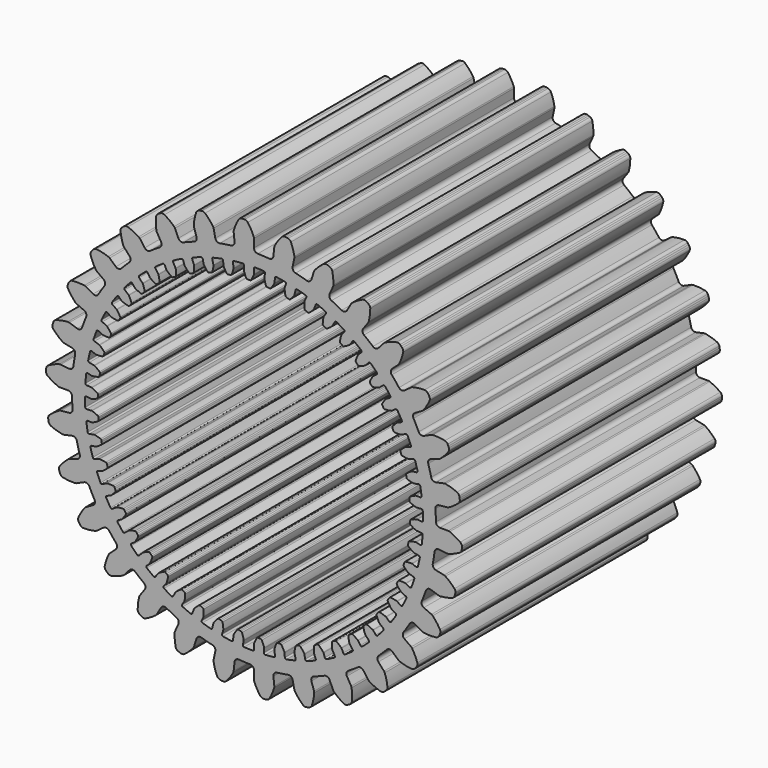
from build123d import *

# Parameters (mm, degrees)
F0_R     = 66.04
F1_DEPTH = 127
F3_DEPTH = 127


with BuildPart() as f1:
    # F0 (on Front) → F1 (new body)
    with BuildSketch(Plane.XZ):
        with BuildLine():
            ThreePointArc((-7.5916945082, 72.2301483765), (-7.9129797204, 71.1242396436), (-8.9162826766, 70.5588711873))
            ThreePointArc((-8.9162826766, 70.5588711873), (-11.1256191537, 70.2443947831), (-13.3240015601, 69.8607570989))
            ThreePointArc((-13.3240015601, 69.8607570989), (-14.4529078355, 70.0884167893), (-15.1002128228, 71.0409159056))
            Line((-15.1002128228, 71.0409159056), (-15.7827713559, 74.2521013318))
            ThreePointArc((-15.7827713559, 74.2521013318), (-15.8703202205, 74.5300140124), (-16.0091602546, 74.7861852573))
            ThreePointArc((-16.0091602546, 74.7861852573), (-17.4478816811, 76.6612354929), (-19.1077086991, 78.3437059976))
            ThreePointArc((-19.1077086991, 78.3437059976), (-19.7318549172, 78.6808116334), (-20.4409902851, 78.6988599396))
            Line((-20.4409902851, 78.6988599396), (-21.0524695561, 78.5688860082))
            Line((-21.0524695561, 78.5688860082), (-21.6470131044, 78.3757070991))
            ThreePointArc((-21.6470131044, 78.3757070991), (-22.2521181946, 78.0055091235), (-22.6240918573, 77.4014939701))
            ThreePointArc((-22.6240918573, 77.4014939701), (-23.2203089684, 75.1145182629), (-23.5287531549, 72.7713164122))
            ThreePointArc((-23.5287531549, 72.7713164122), (-23.520906529, 72.4800455894), (-23.4577697296, 72.1955917156))
            Line((-23.4577697296, 72.1955917156), (-22.4432900457, 69.0733442938))
            ThreePointArc((-22.4432900457, 69.0733442938), (-22.5276230506, 67.9248033683), (-23.3914547183, 67.1631911553))
            ThreePointArc((-23.3914547183, 67.1631911553), (-25.4871285717, 66.3962399325), (-27.5577082884, 65.5639162489))
            ThreePointArc((-27.5577082884, 65.5639162489), (-28.7092783643, 65.5518882164), (-29.5404738864, 66.3489906673))
            Line((-29.5404738864, 66.3489906673), (-30.8757598693, 69.3480920887))
            ThreePointArc((-30.8757598693, 69.3480920887), (-31.0191768766, 69.601729278), (-31.2082439195, 69.8234361003))
            ThreePointArc((-31.2082439195, 69.8234361003), (-33.0053706957, 71.3583849852), (-34.9787317984, 72.6589920309))
            ThreePointArc((-34.9787317984, 72.6589920309), (-35.6593271269, 72.8589638042), (-36.3567186394, 72.7291801782))
            Line((-36.3567186394, 72.7291801782), (-36.9278125215, 72.4749128))
            Line((-36.9278125215, 72.4749128), (-37.4691997131, 72.1623427591))
            ThreePointArc((-37.4691997131, 72.1623427591), (-37.9841133183, 71.6744260751), (-38.2223766521, 71.0062724288))
            ThreePointArc((-38.2223766521, 71.0062724288), (-38.3300760027, 68.6453121202), (-38.144600885, 66.2891856996))
            ThreePointArc((-38.144600885, 66.2891856996), (-38.0763671175, 66.0059112483), (-37.9554687227, 65.7408002529))
            Line((-37.9554687227, 65.7408002529), (-36.3140061133, 62.8977036147))
            ThreePointArc((-36.3140061133, 62.8977036147), (-36.1577011539, 61.7567272465), (-36.8443079442, 60.832157385))
            ThreePointArc((-36.8443079442, 60.832157385), (-38.7347281703, 59.6462507923), (-40.587010928, 58.4016176482))
            ThreePointArc((-40.587010928, 58.4016176482), (-41.7109156662, 58.1504275755), (-42.6896744902, 58.7572961591))
            Line((-42.6896744902, 58.7572961591), (-44.6193295182, 61.4132384523))
            ThreePointArc((-44.6193295182, 61.4132384523), (-44.8123466566, 61.631514988), (-45.0433775713, 61.8090677358))
            ThreePointArc((-45.0433775713, 61.8090677358), (-47.1203666337, 62.9368306381), (-49.3210164716, 63.7987314559))
            ThreePointArc((-49.3210164716, 63.7987314559), (-50.0283156288, 63.8528296407), (-50.6834839304, 63.5808862498))
            Line((-50.6834839304, 63.5808862498), (-51.1892328803, 63.2134381291))
            Line((-51.1892328803, 63.2134381291), (-51.6538024972, 62.7951377672))
            ThreePointArc((-51.6538024972, 62.7951377672), (-52.0560204219, 62.2108266751), (-52.1501601759, 61.5077360565))
            ThreePointArc((-52.1501601759, 61.5077360565), (-51.7646347876, 59.1759764411), (-51.0933465183, 56.9098994811))
            ThreePointArc((-51.0933465183, 56.9098994811), (-50.9677077523, 56.6470018542), (-50.7943316022, 56.4128203598))
            Line((-50.7943316022, 56.4128203598), (-48.5976258599, 53.973131471))
            ThreePointArc((-48.5976258599, 53.973131471), (-48.2075142129, 52.8895858023), (-48.6868881143, 51.8424664319))
            ThreePointArc((-48.6868881143, 51.8424664319), (-50.289434278, 50.289434278), (-51.8424664319, 48.6868881143))
            ThreePointArc((-51.8424664319, 48.6868881143), (-52.8895858023, 48.2075142129), (-53.973131471, 48.5976258599))
            Line((-53.973131471, 48.5976258599), (-56.4128203598, 50.7943316022))
            ThreePointArc((-56.4128203598, 50.7943316022), (-56.6470018542, 50.9677077523), (-56.9098994811, 51.0933465183))
            ThreePointArc((-56.9098994811, 51.0933465183), (-59.1759764411, 51.7646347876), (-61.5077360565, 52.1501601759))
            ThreePointArc((-61.5077360565, 52.1501601759), (-62.2108266751, 52.0560204219), (-62.7951377672, 51.6538024972))
            Line((-62.7951377672, 51.6538024972), (-63.2134381291, 51.1892328803))
            Line((-63.2134381291, 51.1892328803), (-63.5808862498, 50.6834839304))
            ThreePointArc((-63.5808862498, 50.6834839304), (-63.8528296407, 50.0283156288), (-63.7987314559, 49.3210164716))
            ThreePointArc((-63.7987314559, 49.3210164716), (-62.9368306381, 47.1203666337), (-61.8090677358, 45.0433775713))
            ThreePointArc((-61.8090677358, 45.0433775713), (-61.631514988, 44.8123466566), (-61.4132384523, 44.6193295182))
            Line((-61.4132384523, 44.6193295182), (-58.7572961591, 42.6896744902))
            ThreePointArc((-58.7572961591, 42.6896744902), (-58.1504275755, 41.7109156662), (-58.4016176482, 40.587010928))
            ThreePointArc((-58.4016176482, 40.587010928), (-59.6462507923, 38.7347281703), (-60.832157385, 36.8443079442))
            ThreePointArc((-60.832157385, 36.8443079442), (-61.7567272465, 36.1577011539), (-62.8977036147, 36.3140061133))
            Line((-62.8977036147, 36.3140061133), (-65.7408002529, 37.9554687227))
            ThreePointArc((-65.7408002529, 37.9554687227), (-66.0059112483, 38.0763671175), (-66.2891856996, 38.144600885))
            ThreePointArc((-66.2891856996, 38.144600885), (-68.6453121202, 38.3300760027), (-71.0062724288, 38.2223766521))
            ThreePointArc((-71.0062724288, 38.2223766521), (-71.6744260751, 37.9841133183), (-72.1623427591, 37.4691997131))
            Line((-72.1623427591, 37.4691997131), (-72.4749128, 36.9278125215))
            Line((-72.4749128, 36.9278125215), (-72.7291801782, 36.3567186394))
            ThreePointArc((-72.7291801782, 36.3567186394), (-72.8589638042, 35.6593271269), (-72.6589920309, 34.9787317984))
            ThreePointArc((-72.6589920309, 34.9787317984), (-71.3583849852, 33.0053706957), (-69.8234361003, 31.2082439195))
            ThreePointArc((-69.8234361003, 31.2082439195), (-69.601729278, 31.0191768766), (-69.3480920887, 30.8757598693))
            Line((-69.3480920887, 30.8757598693), (-66.3489906673, 29.5404738864))
            ThreePointArc((-66.3489906673, 29.5404738864), (-65.5518882164, 28.7092783643), (-65.5639162489, 27.5577082884))
            ThreePointArc((-65.5639162489, 27.5577082884), (-66.3962399325, 25.4871285717), (-67.1631911553, 23.3914547183))
            ThreePointArc((-67.1631911553, 23.3914547183), (-67.9248033683, 22.5276230506), (-69.0733442938, 22.4432900457))
            Line((-69.0733442938, 22.4432900457), (-72.1955917156, 23.4577697296))
            ThreePointArc((-72.1955917156, 23.4577697296), (-72.4800455894, 23.520906529), (-72.7713164122, 23.5287531548))
            ThreePointArc((-72.7713164122, 23.5287531548), (-75.1145182629, 23.2203089684), (-77.4014939701, 22.6240918573))
            ThreePointArc((-77.4014939701, 22.6240918573), (-78.0055091235, 22.2521181946), (-78.3757070991, 21.6470131044))
            Line((-78.3757070991, 21.6470131044), (-78.5688860082, 21.0524695561))
            Line((-78.5688860082, 21.0524695561), (-78.6988599396, 20.4409902851))
            ThreePointArc((-78.6988599396, 20.4409902851), (-78.6808116334, 19.7318549172), (-78.3437059976, 19.1077086991))
            ThreePointArc((-78.3437059976, 19.1077086991), (-76.6612354929, 17.4478816811), (-74.7861852573, 16.0091602546))
            ThreePointArc((-74.7861852573, 16.0091602546), (-74.5300140124, 15.8703202205), (-74.2521013318, 15.7827713559))
            Line((-74.2521013318, 15.7827713559), (-71.0409159056, 15.1002128228))
            ThreePointArc((-71.0409159056, 15.1002128228), (-70.0884167893, 14.4529078355), (-69.8607570989, 13.3240015601))
            ThreePointArc((-69.8607570989, 13.3240015601), (-70.2443947831, 11.1256191537), (-70.5588711873, 8.9162826766))
            ThreePointArc((-70.5588711873, 8.9162826766), (-71.1242396436, 7.9129797204), (-72.2301483765, 7.5916945082))
            Line((-72.2301483765, 7.5916945082), (-75.4950893875, 7.9348536364))
            ThreePointArc((-75.4950893875, 7.9348536364), (-75.7864541404, 7.9374694594), (-76.0729914021, 7.8845860084))
            ThreePointArc((-76.0729914021, 7.8845860084), (-78.300859518, 7.0957030087), (-80.4138988113, 6.0370256858))
            ThreePointArc((-80.4138988113, 6.0370256858), (-80.9273771113, 5.5475987283), (-81.1636769505, 4.8787481491))
            Line((-81.1636769505, 4.8787481491), (-81.2290218826, 4.2570326502))
            Line((-81.2290218826, 4.2570326502), (-81.2290218826, 3.6318925685))
            ThreePointArc((-81.2290218826, 3.6318925685), (-81.0639304418, 2.9420059637), (-80.6044240774, 2.4015870407))
            ThreePointArc((-80.6044240774, 2.4015870407), (-78.6136221482, 1.1278365127), (-76.4804192545, 0.1103994662))
            ThreePointArc((-76.4804192545, 0.1103994662), (-76.2009794998, 0.0278544166), (-75.9109374455, 0))
            Line((-75.9109374455, 0), (-72.6280122267, 0))
            ThreePointArc((-72.6280122267, 0), (-71.561745227, -0.4351241185), (-71.1043476345, -1.492027972))
            ThreePointArc((-71.1043476345, -1.492027972), (-71.0225325117, -3.722133208), (-70.8707899695, -5.9485737032))
            ThreePointArc((-70.8707899695, -5.9485737032), (-71.2152053544, -7.0474987943), (-72.2301483765, -7.5916945082))
            Line((-72.2301483765, -7.5916945082), (-75.4950893875, -7.9348536364))
            ThreePointArc((-75.4950893875, -7.9348536364), (-75.7806309817, -7.9928731138), (-76.049911629, -8.1041753811))
            ThreePointArc((-76.049911629, -8.1041753811), (-78.0650774831, -9.3390192214), (-79.9118304058, -10.813887477))
            ThreePointArc((-79.9118304058, -10.813887477), (-80.3123303867, -11.3993774227), (-80.4044046526, -12.1027415111))
            Line((-80.4044046526, -12.1027415111), (-80.3390597205, -12.72445701))
            Line((-80.3390597205, -12.72445701), (-80.2090857892, -13.3359362811))
            ThreePointArc((-80.2090857892, -13.3359362811), (-79.904166502, -13.9764227678), (-79.3423420421, -14.4094954956))
            ThreePointArc((-79.3423420421, -14.4094954956), (-77.1302162855, -15.2415005232), (-74.8320919366, -15.7931863087))
            ThreePointArc((-74.8320919366, -15.7931863087), (-74.5415965301, -15.815828759), (-74.2521013318, -15.7827713559))
            Line((-74.2521013318, -15.7827713559), (-71.0409159056, -15.1002128228))
            ThreePointArc((-71.0409159056, -15.1002128228), (-69.9074820069, -15.3041390605), (-69.240336982, -16.2428487223))
            ThreePointArc((-69.240336982, -16.2428487223), (-68.6966447657, -18.4072104877), (-68.0853151542, -20.5534488677))
            ThreePointArc((-68.0853151542, -20.5534488677), (-68.1937248628, -21.699967794), (-69.0733442938, -22.4432900457))
            Line((-69.0733442938, -22.4432900457), (-72.1955917156, -23.4577697296))
            ThreePointArc((-72.1955917156, -23.4577697296), (-72.4628306132, -23.5738887778), (-72.7030857898, -23.7387454183))
            ThreePointArc((-72.7030857898, -23.7387454183), (-74.4174769643, -25.3655814979), (-75.917231552, -27.1921818662))
            ThreePointArc((-75.917231552, -27.1921818662), (-76.1872494429, -27.8481460801), (-76.1310740483, -28.5552832919))
            Line((-76.1310740483, -28.5552832919), (-75.9378951392, -29.1498268402))
            Line((-75.9378951392, -29.1498268402), (-75.6836277609, -29.7209207222))
            ThreePointArc((-75.6836277609, -29.7209207222), (-75.2522070634, -30.284014758), (-74.6126189328, -30.5908139342))
            ThreePointArc((-74.6126189328, -30.5908139342), (-72.2758498594, -30.9447108494), (-69.9132431169, -31.0065340577))
            ThreePointArc((-69.9132431169, -31.0065340577), (-69.6243881018, -30.9682843251), (-69.3480920887, -30.8757598693))
            Line((-69.3480920887, -30.8757598693), (-66.3489906673, -29.5404738864))
            ThreePointArc((-66.3489906673, -29.5404738864), (-65.1979263698, -29.5042896882), (-64.3501913514, -30.2837790415))
            ThreePointArc((-64.3501913514, -30.2837790415), (-63.3683840003, -32.2878043415), (-62.324185357, -34.2600396903))
            ThreePointArc((-62.324185357, -34.2600396903), (-62.191851365, -35.4040440731), (-62.8977036147, -36.3140061133))
            Line((-62.8977036147, -36.3140061133), (-65.7408002529, -37.9554687227))
            ThreePointArc((-65.7408002529, -37.9554687227), (-65.9780568318, -38.1246123823), (-66.1787862334, -38.3358183696))
            ThreePointArc((-66.1787862334, -38.3358183696), (-67.5174756075, -40.2835461454), (-68.6046853881, -42.3820474253))
            ThreePointArc((-68.6046853881, -42.3820474253), (-68.7324201114, -43.0798171236), (-68.5304501906, -43.7598221694))
            Line((-68.5304501906, -43.7598221694), (-68.2178801498, -44.3012093611))
            Line((-68.2178801498, -44.3012093611), (-67.8504320291, -44.806958311))
            ThreePointArc((-67.8504320291, -44.806958311), (-67.3113650759, -45.2680499844), (-66.621966345, -45.4351670129))
            ThreePointArc((-66.621966345, -45.4351670129), (-64.2626819764, -45.2954888223), (-61.9388500919, -44.8647474826))
            ThreePointArc((-61.9388500919, -44.8647474826), (-61.6642598186, -44.7672772638), (-61.4132384523, -44.6193295182))
            Line((-61.4132384523, -44.6193295182), (-58.7572961591, -42.6896744902))
            ThreePointArc((-58.7572961591, -42.6896744902), (-57.638908496, -42.4149612793), (-56.6476335723, -43.0011628989))
            ThreePointArc((-56.6476335723, -43.0011628989), (-55.2706207788, -44.7572662115), (-53.8391895952, -46.4693023806))
            ThreePointArc((-53.8391895952, -46.4693023806), (-53.4718955328, -47.5607937387), (-53.973131471, -48.5976258599))
            Line((-53.973131471, -48.5976258599), (-56.4128203598, -50.7943316022))
            ThreePointArc((-56.4128203598, -50.7943316022), (-56.6097253689, -51.0091074834), (-56.7621561576, -51.2574321024))
            ThreePointArc((-56.7621561576, -51.2574321024), (-57.6666365818, -53.4409265245), (-58.293785271, -55.7196141403))
            ThreePointArc((-58.293785271, -55.7196141403), (-58.2736542063, -56.4286934388), (-57.934716814, -57.0518468352))
            Line((-57.934716814, -57.0518468352), (-57.5164164521, -57.5164164521))
            Line((-57.5164164521, -57.5164164521), (-57.0518468352, -57.934716814))
            ThreePointArc((-57.0518468352, -57.934716814), (-56.4286934388, -58.2736542063), (-55.7196141403, -58.293785271))
            ThreePointArc((-55.7196141403, -58.293785271), (-53.4409265245, -57.6666365818), (-51.2574321024, -56.7621561576))
            ThreePointArc((-51.2574321024, -56.7621561576), (-51.0091074834, -56.6097253689), (-50.7943316022, -56.4128203598))
            Line((-50.7943316022, -56.4128203598), (-48.5976258599, -53.973131471))
            ThreePointArc((-48.5976258599, -53.973131471), (-47.5607937387, -53.4718955328), (-46.4693023806, -53.8391895952))
            ThreePointArc((-46.4693023806, -53.8391895952), (-44.7572662115, -55.2706207788), (-43.0011628989, -56.6476335723))
            ThreePointArc((-43.0011628989, -56.6476335723), (-42.4149612793, -57.638908496), (-42.6896744902, -58.7572961591))
            Line((-42.6896744902, -58.7572961591), (-44.6193295182, -61.4132384523))
            ThreePointArc((-44.6193295182, -61.4132384523), (-44.7672772638, -61.6642598186), (-44.8647474826, -61.9388500919))
            ThreePointArc((-44.8647474826, -61.9388500919), (-45.2954888223, -64.2626819764), (-45.4351670129, -66.621966345))
            ThreePointArc((-45.4351670129, -66.621966345), (-45.2680499844, -67.3113650759), (-44.806958311, -67.8504320291))
            Line((-44.806958311, -67.8504320291), (-44.3012093611, -68.2178801498))
            Line((-44.3012093611, -68.2178801498), (-43.7598221694, -68.5304501906))
            ThreePointArc((-43.7598221694, -68.5304501906), (-43.0798171236, -68.7324201114), (-42.3820474253, -68.6046853881))
            ThreePointArc((-42.3820474253, -68.6046853881), (-40.2835461454, -67.5174756075), (-38.3358183696, -66.1787862334))
            ThreePointArc((-38.3358183696, -66.1787862334), (-38.1246123823, -65.9780568318), (-37.9554687227, -65.7408002529))
            Line((-37.9554687227, -65.7408002529), (-36.3140061133, -62.8977036147))
            ThreePointArc((-36.3140061133, -62.8977036147), (-35.4040440731, -62.191851365), (-34.2600396903, -62.324185357))
            ThreePointArc((-34.2600396903, -62.324185357), (-32.2878043415, -63.3683840003), (-30.2837790415, -64.3501913514))
            ThreePointArc((-30.2837790415, -64.3501913514), (-29.5042896882, -65.1979263698), (-29.5404738864, -66.3489906673))
            Line((-29.5404738864, -66.3489906673), (-30.8757598693, -69.3480920887))
            ThreePointArc((-30.8757598693, -69.3480920887), (-30.9682843251, -69.6243881018), (-31.0065340577, -69.9132431169))
            ThreePointArc((-31.0065340577, -69.9132431169), (-30.9447108494, -72.2758498594), (-30.5908139342, -74.6126189328))
            ThreePointArc((-30.5908139342, -74.6126189328), (-30.284014758, -75.2522070634), (-29.7209207222, -75.6836277609))
            Line((-29.7209207222, -75.6836277609), (-29.1498268402, -75.9378951392))
            Line((-29.1498268402, -75.9378951392), (-28.5552832919, -76.1310740483))
            ThreePointArc((-28.5552832919, -76.1310740483), (-27.8481460801, -76.1872494429), (-27.1921818662, -75.917231552))
            ThreePointArc((-27.1921818662, -75.917231552), (-25.3655814979, -74.4174769643), (-23.7387454183, -72.7030857898))
            ThreePointArc((-23.7387454183, -72.7030857898), (-23.5738887778, -72.4628306132), (-23.4577697296, -72.1955917156))
            Line((-23.4577697296, -72.1955917156), (-22.4432900457, -69.0733442938))
            ThreePointArc((-22.4432900457, -69.0733442938), (-21.699967794, -68.1937248628), (-20.5534488677, -68.0853151542))
            ThreePointArc((-20.5534488677, -68.0853151542), (-18.4072104877, -68.6966447657), (-16.2428487223, -69.240336982))
            ThreePointArc((-16.2428487223, -69.240336982), (-15.3041390605, -69.9074820069), (-15.1002128228, -71.0409159056))
            Line((-15.1002128228, -71.0409159056), (-15.7827713559, -74.2521013318))
            ThreePointArc((-15.7827713559, -74.2521013318), (-15.815828759, -74.5415965301), (-15.7931863087, -74.8320919366))
            ThreePointArc((-15.7931863087, -74.8320919366), (-15.2415005232, -77.1302162855), (-14.4094954956, -79.3423420421))
            ThreePointArc((-14.4094954956, -79.3423420421), (-13.9764227678, -79.904166502), (-13.3359362811, -80.2090857892))
            Line((-13.3359362811, -80.2090857892), (-12.72445701, -80.3390597205))
            Line((-12.72445701, -80.3390597205), (-12.1027415111, -80.4044046526))
            ThreePointArc((-12.1027415111, -80.4044046526), (-11.3993774227, -80.3123303867), (-10.813887477, -79.9118304058))
            ThreePointArc((-10.813887477, -79.9118304058), (-9.3390192214, -78.0650774831), (-8.1041753811, -76.049911629))
            ThreePointArc((-8.1041753811, -76.049911629), (-7.9928731138, -75.7806309817), (-7.9348536364, -75.4950893875))
            Line((-7.9348536364, -75.4950893875), (-7.5916945082, -72.2301483765))
            ThreePointArc((-7.5916945082, -72.2301483765), (-7.0474987943, -71.2152053544), (-5.9485737032, -70.8707899695))
            ThreePointArc((-5.9485737032, -70.8707899695), (-3.722133208, -71.0225325117), (-1.492027972, -71.1043476345))
            ThreePointArc((-1.492027972, -71.1043476345), (-0.4351241185, -71.561745227), (0, -72.6280122267))
            Line((0, -72.6280122267), (0, -75.9109374455))
            ThreePointArc((0, -75.9109374455), (0.0278544166, -76.2009794998), (0.1103994662, -76.4804192545))
            ThreePointArc((0.1103994662, -76.4804192545), (1.1278365127, -78.6136221482), (2.4015870407, -80.6044240774))
            ThreePointArc((2.4015870407, -80.6044240774), (2.9420059637, -81.0639304418), (3.6318925685, -81.2290218826))
            Line((3.6318925685, -81.2290218826), (4.2570326502, -81.2290218826))
            Line((4.2570326502, -81.2290218826), (4.8787481491, -81.1636769505))
            ThreePointArc((4.8787481491, -81.1636769505), (5.5475987283, -80.9273771113), (6.0370256858, -80.4138988113))
            ThreePointArc((6.0370256858, -80.4138988113), (7.0957030087, -78.300859518), (7.8845860084, -76.0729914021))
            ThreePointArc((7.8845860084, -76.0729914021), (7.9374694594, -75.7864541404), (7.9348536364, -75.4950893875))
            Line((7.9348536364, -75.4950893875), (7.5916945082, -72.2301483765))
            ThreePointArc((7.5916945082, -72.2301483765), (7.9129797204, -71.1242396436), (8.9162826766, -70.5588711873))
            ThreePointArc((8.9162826766, -70.5588711873), (11.1256191537, -70.2443947831), (13.3240015601, -69.8607570989))
            ThreePointArc((13.3240015601, -69.8607570989), (14.4529078355, -70.0884167893), (15.1002128228, -71.0409159056))
            Line((15.1002128228, -71.0409159056), (15.7827713559, -74.2521013318))
            ThreePointArc((15.7827713559, -74.2521013318), (15.8703202205, -74.5300140124), (16.0091602546, -74.7861852573))
            ThreePointArc((16.0091602546, -74.7861852573), (17.4478816811, -76.6612354929), (19.1077086991, -78.3437059976))
            ThreePointArc((19.1077086991, -78.3437059976), (19.7318549172, -78.6808116334), (20.4409902851, -78.6988599396))
            Line((20.4409902851, -78.6988599396), (21.0524695561, -78.5688860082))
            Line((21.0524695561, -78.5688860082), (21.6470131044, -78.3757070991))
            ThreePointArc((21.6470131044, -78.3757070991), (22.2521181946, -78.0055091235), (22.6240918573, -77.4014939701))
            ThreePointArc((22.6240918573, -77.4014939701), (23.2203089684, -75.1145182629), (23.5287531548, -72.7713164122))
            ThreePointArc((23.5287531548, -72.7713164122), (23.520906529, -72.4800455894), (23.4577697296, -72.1955917156))
            Line((23.4577697296, -72.1955917156), (22.4432900457, -69.0733442938))
            ThreePointArc((22.4432900457, -69.0733442938), (22.5276230506, -67.9248033683), (23.3914547183, -67.1631911553))
            ThreePointArc((23.3914547183, -67.1631911553), (25.4871285717, -66.3962399325), (27.5577082884, -65.5639162489))
            ThreePointArc((27.5577082884, -65.5639162489), (28.7092783643, -65.5518882164), (29.5404738864, -66.3489906673))
            Line((29.5404738864, -66.3489906673), (30.8757598693, -69.3480920887))
            ThreePointArc((30.8757598693, -69.3480920887), (31.0191768766, -69.601729278), (31.2082439195, -69.8234361003))
            ThreePointArc((31.2082439195, -69.8234361003), (33.0053706957, -71.3583849852), (34.9787317984, -72.6589920309))
            ThreePointArc((34.9787317984, -72.6589920309), (35.6593271269, -72.8589638042), (36.3567186394, -72.7291801782))
            Line((36.3567186394, -72.7291801782), (36.9278125215, -72.4749128))
            Line((36.9278125215, -72.4749128), (37.4691997131, -72.1623427591))
            ThreePointArc((37.4691997131, -72.1623427591), (37.9841133183, -71.6744260751), (38.2223766521, -71.0062724288))
            ThreePointArc((38.2223766521, -71.0062724288), (38.3300760027, -68.6453121202), (38.144600885, -66.2891856996))
            ThreePointArc((38.144600885, -66.2891856996), (38.0763671175, -66.0059112483), (37.9554687227, -65.7408002529))
            Line((37.9554687227, -65.7408002529), (36.3140061133, -62.8977036147))
            ThreePointArc((36.3140061133, -62.8977036147), (36.1577011539, -61.7567272465), (36.8443079442, -60.832157385))
            ThreePointArc((36.8443079442, -60.832157385), (38.7347281703, -59.6462507923), (40.587010928, -58.4016176482))
            ThreePointArc((40.587010928, -58.4016176482), (41.7109156662, -58.1504275755), (42.6896744902, -58.7572961591))
            Line((42.6896744902, -58.7572961591), (44.6193295182, -61.4132384523))
            ThreePointArc((44.6193295182, -61.4132384523), (44.8123466566, -61.631514988), (45.0433775713, -61.8090677358))
            ThreePointArc((45.0433775713, -61.8090677358), (47.1203666337, -62.9368306381), (49.3210164716, -63.7987314559))
            ThreePointArc((49.3210164716, -63.7987314559), (50.0283156288, -63.8528296407), (50.6834839304, -63.5808862498))
            Line((50.6834839304, -63.5808862498), (51.1892328803, -63.2134381291))
            Line((51.1892328803, -63.2134381291), (51.6538024972, -62.7951377672))
            ThreePointArc((51.6538024972, -62.7951377672), (52.0560204219, -62.2108266751), (52.1501601759, -61.5077360565))
            ThreePointArc((52.1501601759, -61.5077360565), (51.7646347876, -59.1759764411), (51.0933465183, -56.9098994811))
            ThreePointArc((51.0933465183, -56.9098994811), (50.9677077523, -56.6470018542), (50.7943316022, -56.4128203598))
            Line((50.7943316022, -56.4128203598), (48.5976258599, -53.973131471))
            ThreePointArc((48.5976258599, -53.973131471), (48.2075142129, -52.8895858023), (48.6868881143, -51.8424664319))
            ThreePointArc((48.6868881143, -51.8424664319), (50.289434278, -50.289434278), (51.8424664319, -48.6868881143))
            ThreePointArc((51.8424664319, -48.6868881143), (52.8895858023, -48.2075142129), (53.973131471, -48.5976258599))
            Line((53.973131471, -48.5976258599), (56.4128203598, -50.7943316022))
            ThreePointArc((56.4128203598, -50.7943316022), (56.6470018542, -50.9677077523), (56.9098994811, -51.0933465183))
            ThreePointArc((56.9098994811, -51.0933465183), (59.1759764411, -51.7646347876), (61.5077360565, -52.1501601759))
            ThreePointArc((61.5077360565, -52.1501601759), (62.2108266751, -52.0560204219), (62.7951377672, -51.6538024972))
            Line((62.7951377672, -51.6538024972), (63.2134381291, -51.1892328803))
            Line((63.2134381291, -51.1892328803), (63.5808862498, -50.6834839304))
            ThreePointArc((63.5808862498, -50.6834839304), (63.8528296407, -50.0283156288), (63.7987314559, -49.3210164716))
            ThreePointArc((63.7987314559, -49.3210164716), (62.9368306381, -47.1203666337), (61.8090677358, -45.0433775713))
            ThreePointArc((61.8090677358, -45.0433775713), (61.631514988, -44.8123466566), (61.4132384523, -44.6193295182))
            Line((61.4132384523, -44.6193295182), (58.7572961591, -42.6896744902))
            ThreePointArc((58.7572961591, -42.6896744902), (58.1504275755, -41.7109156662), (58.4016176482, -40.587010928))
            ThreePointArc((58.4016176482, -40.587010928), (59.6462507923, -38.7347281703), (60.832157385, -36.8443079442))
            ThreePointArc((60.832157385, -36.8443079442), (61.7567272465, -36.1577011539), (62.8977036147, -36.3140061133))
            Line((62.8977036147, -36.3140061133), (65.7408002529, -37.9554687227))
            ThreePointArc((65.7408002529, -37.9554687227), (66.0059112483, -38.0763671175), (66.2891856996, -38.144600885))
            ThreePointArc((66.2891856996, -38.144600885), (68.6453121202, -38.3300760027), (71.0062724288, -38.2223766521))
            ThreePointArc((71.0062724288, -38.2223766521), (71.6744260751, -37.9841133183), (72.1623427591, -37.4691997131))
            Line((72.1623427591, -37.4691997131), (72.4749128, -36.9278125215))
            Line((72.4749128, -36.9278125215), (72.7291801782, -36.3567186394))
            ThreePointArc((72.7291801782, -36.3567186394), (72.8589638042, -35.6593271269), (72.6589920309, -34.9787317984))
            ThreePointArc((72.6589920309, -34.9787317984), (71.3583849852, -33.0053706957), (69.8234361003, -31.2082439195))
            ThreePointArc((69.8234361003, -31.2082439195), (69.601729278, -31.0191768766), (69.3480920887, -30.8757598693))
            Line((69.3480920887, -30.8757598693), (66.3489906673, -29.5404738864))
            ThreePointArc((66.3489906673, -29.5404738864), (65.5518882164, -28.7092783643), (65.5639162489, -27.5577082884))
            ThreePointArc((65.5639162489, -27.5577082884), (66.3962399325, -25.4871285717), (67.1631911553, -23.3914547183))
            ThreePointArc((67.1631911553, -23.3914547183), (67.9248033683, -22.5276230506), (69.0733442938, -22.4432900457))
            Line((69.0733442938, -22.4432900457), (72.1955917156, -23.4577697296))
            ThreePointArc((72.1955917156, -23.4577697296), (72.4800455894, -23.520906529), (72.7713164122, -23.5287531548))
            ThreePointArc((72.7713164122, -23.5287531548), (75.1145182629, -23.2203089684), (77.4014939701, -22.6240918573))
            ThreePointArc((77.4014939701, -22.6240918573), (78.0055091235, -22.2521181946), (78.3757070991, -21.6470131044))
            Line((78.3757070991, -21.6470131044), (78.5688860082, -21.0524695561))
            Line((78.5688860082, -21.0524695561), (78.6988599396, -20.4409902851))
            ThreePointArc((78.6988599396, -20.4409902851), (78.6808116334, -19.7318549172), (78.3437059976, -19.1077086991))
            ThreePointArc((78.3437059976, -19.1077086991), (76.6612354929, -17.4478816811), (74.7861852573, -16.0091602546))
            ThreePointArc((74.7861852573, -16.0091602546), (74.5300140124, -15.8703202205), (74.2521013318, -15.7827713559))
            Line((74.2521013318, -15.7827713559), (71.0409159056, -15.1002128228))
            ThreePointArc((71.0409159056, -15.1002128228), (70.0884167893, -14.4529078355), (69.8607570989, -13.3240015601))
            ThreePointArc((69.8607570989, -13.3240015601), (70.2443947831, -11.1256191537), (70.5588711873, -8.9162826766))
            ThreePointArc((70.5588711873, -8.9162826766), (71.1242396436, -7.9129797204), (72.2301483765, -7.5916945082))
            Line((72.2301483765, -7.5916945082), (75.4950893875, -7.9348536364))
            ThreePointArc((75.4950893875, -7.9348536364), (75.7864541404, -7.9374694594), (76.0729914021, -7.8845860084))
            ThreePointArc((76.0729914021, -7.8845860084), (78.300859518, -7.0957030087), (80.4138988113, -6.0370256858))
            ThreePointArc((80.4138988113, -6.0370256858), (80.9273771113, -5.5475987283), (81.1636769505, -4.8787481491))
            Line((81.1636769505, -4.8787481491), (81.2290218826, -4.2570326502))
            Line((81.2290218826, -4.2570326502), (81.2290218826, -3.6318925685))
            ThreePointArc((81.2290218826, -3.6318925685), (81.0639304418, -2.9420059637), (80.6044240774, -2.4015870407))
            ThreePointArc((80.6044240774, -2.4015870407), (78.6136221482, -1.1278365127), (76.4804192545, -0.1103994662))
            ThreePointArc((76.4804192545, -0.1103994662), (76.2009794998, -0.0278544166), (75.9109374455, 0))
            Line((75.9109374455, 0), (72.6280122267, 0))
            ThreePointArc((72.6280122267, 0), (71.561745227, 0.4351241185), (71.1043476345, 1.492027972))
            ThreePointArc((71.1043476345, 1.492027972), (71.0225325117, 3.722133208), (70.8707899695, 5.9485737032))
            ThreePointArc((70.8707899695, 5.9485737032), (71.2152053544, 7.0474987943), (72.2301483765, 7.5916945082))
            Line((72.2301483765, 7.5916945082), (75.4950893875, 7.9348536364))
            ThreePointArc((75.4950893875, 7.9348536364), (75.7806309817, 7.9928731138), (76.049911629, 8.1041753811))
            ThreePointArc((76.049911629, 8.1041753811), (78.0650774831, 9.3390192214), (79.9118304058, 10.813887477))
            ThreePointArc((79.9118304058, 10.813887477), (80.3123303867, 11.3993774227), (80.4044046526, 12.1027415111))
            Line((80.4044046526, 12.1027415111), (80.3390597205, 12.72445701))
            Line((80.3390597205, 12.72445701), (80.2090857892, 13.3359362811))
            ThreePointArc((80.2090857892, 13.3359362811), (79.904166502, 13.9764227678), (79.3423420421, 14.4094954956))
            ThreePointArc((79.3423420421, 14.4094954956), (77.1302162855, 15.2415005232), (74.8320919366, 15.7931863087))
            ThreePointArc((74.8320919366, 15.7931863087), (74.5415965301, 15.815828759), (74.2521013318, 15.7827713559))
            Line((74.2521013318, 15.7827713559), (71.0409159056, 15.1002128228))
            ThreePointArc((71.0409159056, 15.1002128228), (69.9074820069, 15.3041390605), (69.240336982, 16.2428487223))
            ThreePointArc((69.240336982, 16.2428487223), (68.6966447657, 18.4072104877), (68.0853151542, 20.5534488677))
            ThreePointArc((68.0853151542, 20.5534488677), (68.1937248628, 21.699967794), (69.0733442938, 22.4432900457))
            Line((69.0733442938, 22.4432900457), (72.1955917156, 23.4577697296))
            ThreePointArc((72.1955917156, 23.4577697296), (72.4628306132, 23.5738887778), (72.7030857898, 23.7387454183))
            ThreePointArc((72.7030857898, 23.7387454183), (74.4174769643, 25.3655814979), (75.917231552, 27.1921818662))
            ThreePointArc((75.917231552, 27.1921818662), (76.1872494429, 27.8481460801), (76.1310740483, 28.5552832919))
            Line((76.1310740483, 28.5552832919), (75.9378951392, 29.1498268402))
            Line((75.9378951392, 29.1498268402), (75.6836277609, 29.7209207222))
            ThreePointArc((75.6836277609, 29.7209207222), (75.2522070634, 30.284014758), (74.6126189328, 30.5908139342))
            ThreePointArc((74.6126189328, 30.5908139342), (72.2758498594, 30.9447108494), (69.9132431169, 31.0065340577))
            ThreePointArc((69.9132431169, 31.0065340577), (69.6243881018, 30.9682843251), (69.3480920887, 30.8757598693))
            Line((69.3480920887, 30.8757598693), (66.3489906673, 29.5404738864))
            ThreePointArc((66.3489906673, 29.5404738864), (65.1979263698, 29.5042896882), (64.3501913514, 30.2837790415))
            ThreePointArc((64.3501913514, 30.2837790415), (63.3683840003, 32.2878043415), (62.324185357, 34.2600396903))
            ThreePointArc((62.324185357, 34.2600396903), (62.191851365, 35.4040440731), (62.8977036147, 36.3140061133))
            Line((62.8977036147, 36.3140061133), (65.7408002529, 37.9554687227))
            ThreePointArc((65.7408002529, 37.9554687227), (65.9780568318, 38.1246123823), (66.1787862334, 38.3358183696))
            ThreePointArc((66.1787862334, 38.3358183696), (67.5174756075, 40.2835461454), (68.6046853881, 42.3820474253))
            ThreePointArc((68.6046853881, 42.3820474253), (68.7324201114, 43.0798171236), (68.5304501906, 43.7598221694))
            Line((68.5304501906, 43.7598221694), (68.2178801498, 44.3012093611))
            Line((68.2178801498, 44.3012093611), (67.8504320291, 44.806958311))
            ThreePointArc((67.8504320291, 44.806958311), (67.3113650759, 45.2680499844), (66.621966345, 45.4351670129))
            ThreePointArc((66.621966345, 45.4351670129), (64.2626819764, 45.2954888223), (61.9388500919, 44.8647474826))
            ThreePointArc((61.9388500919, 44.8647474826), (61.6642598186, 44.7672772638), (61.4132384523, 44.6193295182))
            Line((61.4132384523, 44.6193295182), (58.7572961591, 42.6896744902))
            ThreePointArc((58.7572961591, 42.6896744902), (57.638908496, 42.4149612793), (56.6476335723, 43.0011628989))
            ThreePointArc((56.6476335723, 43.0011628989), (55.2706207788, 44.7572662115), (53.8391895952, 46.4693023806))
            ThreePointArc((53.8391895952, 46.4693023806), (53.4718955328, 47.5607937387), (53.973131471, 48.5976258599))
            Line((53.973131471, 48.5976258599), (56.4128203598, 50.7943316022))
            ThreePointArc((56.4128203598, 50.7943316022), (56.6097253689, 51.0091074834), (56.7621561576, 51.2574321024))
            ThreePointArc((56.7621561576, 51.2574321024), (57.6666365818, 53.4409265245), (58.293785271, 55.7196141403))
            ThreePointArc((58.293785271, 55.7196141403), (58.2736542063, 56.4286934388), (57.934716814, 57.0518468352))
            Line((57.934716814, 57.0518468352), (57.5164164521, 57.5164164521))
            Line((57.5164164521, 57.5164164521), (57.0518468352, 57.934716814))
            ThreePointArc((57.0518468352, 57.934716814), (56.4286934388, 58.2736542063), (55.7196141403, 58.293785271))
            ThreePointArc((55.7196141403, 58.293785271), (53.4409265245, 57.6666365818), (51.2574321024, 56.7621561576))
            ThreePointArc((51.2574321024, 56.7621561576), (51.0091074834, 56.6097253689), (50.7943316022, 56.4128203598))
            Line((50.7943316022, 56.4128203598), (48.5976258599, 53.973131471))
            ThreePointArc((48.5976258599, 53.973131471), (47.5607937387, 53.4718955328), (46.4693023806, 53.8391895952))
            ThreePointArc((46.4693023806, 53.8391895952), (44.7572662115, 55.2706207788), (43.0011628989, 56.6476335723))
            ThreePointArc((43.0011628989, 56.6476335723), (42.4149612793, 57.638908496), (42.6896744902, 58.7572961591))
            Line((42.6896744902, 58.7572961591), (44.6193295182, 61.4132384523))
            ThreePointArc((44.6193295182, 61.4132384523), (44.7672772638, 61.6642598186), (44.8647474826, 61.9388500919))
            ThreePointArc((44.8647474826, 61.9388500919), (45.2954888223, 64.2626819764), (45.4351670129, 66.621966345))
            ThreePointArc((45.4351670129, 66.621966345), (45.2680499844, 67.3113650759), (44.806958311, 67.8504320291))
            Line((44.806958311, 67.8504320291), (44.3012093611, 68.2178801498))
            Line((44.3012093611, 68.2178801498), (43.7598221694, 68.5304501906))
            ThreePointArc((43.7598221694, 68.5304501906), (43.0798171236, 68.7324201114), (42.3820474253, 68.6046853881))
            ThreePointArc((42.3820474253, 68.6046853881), (40.2835461454, 67.5174756075), (38.3358183696, 66.1787862334))
            ThreePointArc((38.3358183696, 66.1787862334), (38.1246123823, 65.9780568318), (37.9554687227, 65.7408002529))
            Line((37.9554687227, 65.7408002529), (36.3140061133, 62.8977036147))
            ThreePointArc((36.3140061133, 62.8977036147), (35.4040440731, 62.191851365), (34.2600396903, 62.324185357))
            ThreePointArc((34.2600396903, 62.324185357), (32.2878043415, 63.3683840003), (30.2837790415, 64.3501913514))
            ThreePointArc((30.2837790415, 64.3501913514), (29.5042896882, 65.1979263698), (29.5404738864, 66.3489906673))
            Line((29.5404738864, 66.3489906673), (30.8757598693, 69.3480920887))
            ThreePointArc((30.8757598693, 69.3480920887), (30.9682843251, 69.6243881018), (31.0065340577, 69.9132431169))
            ThreePointArc((31.0065340577, 69.9132431169), (30.9447108494, 72.2758498594), (30.5908139342, 74.6126189328))
            ThreePointArc((30.5908139342, 74.6126189328), (30.284014758, 75.2522070634), (29.7209207222, 75.6836277609))
            Line((29.7209207222, 75.6836277609), (29.1498268402, 75.9378951392))
            Line((29.1498268402, 75.9378951392), (28.5552832919, 76.1310740483))
            ThreePointArc((28.5552832919, 76.1310740483), (27.8481460801, 76.1872494429), (27.1921818662, 75.917231552))
            ThreePointArc((27.1921818662, 75.917231552), (25.3655814979, 74.4174769643), (23.7387454183, 72.7030857898))
            ThreePointArc((23.7387454183, 72.7030857898), (23.5738887778, 72.4628306132), (23.4577697296, 72.1955917156))
            Line((23.4577697296, 72.1955917156), (22.4432900457, 69.0733442938))
            ThreePointArc((22.4432900457, 69.0733442938), (21.699967794, 68.1937248628), (20.5534488677, 68.0853151542))
            ThreePointArc((20.5534488677, 68.0853151542), (18.4072104877, 68.6966447657), (16.2428487223, 69.240336982))
            ThreePointArc((16.2428487223, 69.240336982), (15.3041390605, 69.9074820069), (15.1002128228, 71.0409159056))
            Line((15.1002128228, 71.0409159056), (15.7827713559, 74.2521013318))
            ThreePointArc((15.7827713559, 74.2521013318), (15.815828759, 74.5415965301), (15.7931863087, 74.8320919366))
            ThreePointArc((15.7931863087, 74.8320919366), (15.2415005232, 77.1302162855), (14.4094954956, 79.3423420421))
            ThreePointArc((14.4094954956, 79.3423420421), (13.9764227678, 79.904166502), (13.3359362811, 80.2090857892))
            Line((13.3359362811, 80.2090857892), (12.72445701, 80.3390597205))
            Line((12.72445701, 80.3390597205), (12.1027415111, 80.4044046526))
            ThreePointArc((12.1027415111, 80.4044046526), (11.3993774227, 80.3123303867), (10.813887477, 79.9118304058))
            ThreePointArc((10.813887477, 79.9118304058), (9.3390192214, 78.0650774831), (8.1041753811, 76.049911629))
            ThreePointArc((8.1041753811, 76.049911629), (7.9928731138, 75.7806309817), (7.9348536364, 75.4950893875))
            Line((7.9348536364, 75.4950893875), (7.5916945082, 72.2301483765))
            ThreePointArc((7.5916945082, 72.2301483765), (7.0474987943, 71.2152053544), (5.9485737032, 70.8707899695))
            ThreePointArc((5.9485737032, 70.8707899695), (3.722133208, 71.0225325117), (1.492027972, 71.1043476345))
            ThreePointArc((1.492027972, 71.1043476345), (0.4351241185, 71.561745227), (0, 72.6280122267))
            Line((0, 72.6280122267), (0, 75.9109374455))
            ThreePointArc((0, 75.9109374455), (-0.0278544166, 76.2009794998), (-0.1103994662, 76.4804192545))
            ThreePointArc((-0.1103994662, 76.4804192545), (-1.1278365127, 78.6136221482), (-2.4015870407, 80.6044240774))
            ThreePointArc((-2.4015870407, 80.6044240774), (-2.9420059637, 81.0639304418), (-3.6318925685, 81.2290218826))
            Line((-3.6318925685, 81.2290218826), (-4.2570326502, 81.2290218826))
            Line((-4.2570326502, 81.2290218826), (-4.8787481491, 81.1636769505))
            ThreePointArc((-4.8787481491, 81.1636769505), (-5.5475987283, 80.9273771113), (-6.0370256858, 80.4138988113))
            ThreePointArc((-6.0370256858, 80.4138988113), (-7.0957030087, 78.300859518), (-7.8845860084, 76.0729914021))
            ThreePointArc((-7.8845860084, 76.0729914021), (-7.9374694594, 75.7864541404), (-7.9348536364, 75.4950893875))
            Line((-7.9348536364, 75.4950893875), (-7.5916945082, 72.2301483765))
        make_face()
        Circle(F0_R, mode=Mode.SUBTRACT)
    extrude(amount=F1_DEPTH)

    # F2 (on face) → F3 (join)
    with BuildSketch(Plane.XZ.offset(127)):
        with BuildLine():
            Line((-3.8865696855, 65.3526540372), (-3.9879510392, 63.7412435639))
            ThreePointArc((-3.9879510392, 63.7412435639), (-3.9851112222, 63.6469845176), (-3.9648982324, 63.5548744345))
            ThreePointArc((-3.9648982324, 63.5548744345), (-3.5486424942, 62.405553041), (-3.0451883851, 61.2916668416))
            ThreePointArc((-3.0451883851, 61.2916668416), (-2.8673349589, 61.0925059916), (-2.6130468451, 61.0110539163))
            Line((-2.6130468451, 61.0110539163), (-2.074532217, 60.9873144911))
            Line((-2.074532217, 60.9873144911), (-1.5355896138, 60.9771934587))
            ThreePointArc((-1.5355896138, 60.9771934587), (-1.2766888613, 61.0425179242), (-1.086680975, 61.2301182667))
            ThreePointArc((-1.086680975, 61.2301182667), (-0.5192282273, 62.2999268001), (-0.0349750375, 63.4098780455))
            ThreePointArc((-0.0349750375, 63.4098780455), (-0.0088203325, 63.5008582038), (0, 63.595111371))
            Line((0, 63.595111371), (0, 65.5300309782))
            ThreePointArc((0, 65.5300309782), (0.1501847517, 65.890630823), (0.5119379845, 66.0380157144))
            ThreePointArc((0.5119379845, 66.0380157144), (0.255970915, 66.0395039267), (0, 66.04))
            ThreePointArc((0, 66.04), (-1.9260160276, 66.0119084883), (-3.8503935118, 65.9276578516))
            ThreePointArc((-3.8503935118, 65.9276578516), (-4.1390494016, 65.9101651496), (-4.4276259245, 65.8914086105))
            ThreePointArc((-4.4276259245, 65.8914086105), (-4.0351235059, 65.7445267212), (-3.8865696855, 65.3526540372))
        make_face()
        with BuildLine():
            ThreePointArc((8.7846592482, 65.4531233929), (6.3295967263, 65.7359704065), (3.8656705337, 65.9267638469))
            ThreePointArc((3.8656705337, 65.9267638469), (4.2366687713, 65.7318465679), (4.3349365298, 65.3244451864))
            Line((4.3349365298, 65.3244451864), (4.0323913131, 63.7384476189))
            ThreePointArc((4.0323913131, 63.7384476189), (4.0233949463, 63.6445759099), (4.031904096, 63.5506587829))
            ThreePointArc((4.031904096, 63.5506587829), (4.3008293668, 62.3582294542), (4.6607066307, 61.1900270488))
            ThreePointArc((4.6607066307, 61.1900270488), (4.8121961562, 60.9701456965), (5.0542704803, 60.8574651436))
            Line((5.0542704803, 60.8574651436), (5.5855634207, 60.7664191312))
            Line((5.5855634207, 60.7664191312), (6.1189877988, 60.688830487))
            ThreePointArc((6.1189877988, 60.688830487), (6.384034368, 60.7211909811), (6.5960565429, 60.8834977361))
            ThreePointArc((6.5960565429, 60.8834977361), (7.293117319, 61.8737498219), (7.9126658065, 62.9142557521))
            ThreePointArc((7.9126658065, 62.9142557521), (7.9500171113, 63.0012404508), (7.970580947, 63.0936449229))
            Line((7.970580947, 63.0936449229), (8.2130906781, 65.013307111))
            ThreePointArc((8.2130906781, 65.013307111), (8.4072863227, 65.3522403778), (8.7846592482, 65.4531233929))
        make_face()
        with BuildLine():
            ThreePointArc((16.9188411879, 63.8359962158), (14.5185876981, 64.4243138206), (12.0980030582, 64.9224146347))
            ThreePointArc((12.0980030582, 64.9224146347), (12.4416462511, 64.6825359279), (12.4880782065, 64.2660308121))
            Line((12.4880782065, 64.2660308121), (11.9891404457, 62.7304582794))
            ThreePointArc((11.9891404457, 62.7304582794), (11.968449773, 62.6384543206), (11.9651208884, 62.5442112789))
            ThreePointArc((11.9651208884, 62.5442112789), (12.0824745795, 61.3274793379), (12.2930995187, 60.1233839762))
            ThreePointArc((12.2930995187, 60.1233839762), (12.4158360632, 59.886249782), (12.6418789409, 59.7441177911))
            Line((12.6418789409, 59.7441177911), (13.1575713866, 59.5872010415))
            Line((13.1575713866, 59.5872010415), (13.6770651186, 59.4433684048))
            ThreePointArc((13.6770651186, 59.4433684048), (13.9440775617, 59.4422545831), (14.1747703089, 59.5767080761))
            ThreePointArc((14.1747703089, 59.5767080761), (14.9904460485, 60.4717868474), (15.7355191839, 61.4264380623))
            ThreePointArc((15.7355191839, 61.4264380623), (15.7834780361, 61.5080555009), (15.8154610711, 61.597154004))
            Line((15.8154610711, 61.597154004), (16.2966560099, 63.4712845537))
            ThreePointArc((16.2966560099, 63.4712845537), (16.5317999661, 63.7832060623), (16.9188411879, 63.8359962158))
        make_face()
        with BuildLine():
            ThreePointArc((24.7862028953, 61.2121372445), (22.4786118689, 62.0966473205), (20.1395428476, 62.894200161))
            ThreePointArc((20.1395428476, 62.894200161), (20.4504115372, 62.6131430569), (20.4442754299, 62.1941027412))
            Line((20.4442754299, 62.1941027412), (19.7568136714, 60.7331721395))
            ThreePointArc((19.7568136714, 60.7331721395), (19.7247549972, 60.6444868882), (19.7096405767, 60.551404201))
            ThreePointArc((19.7096405767, 60.551404201), (19.6735719504, 59.3295582372), (19.7316228838, 58.1085592223))
            ThreePointArc((19.7316228838, 58.1085592223), (19.8236708186, 57.8579119341), (20.0301174187, 57.6885700117))
            Line((20.0301174187, 57.6885700117), (20.5220765918, 57.4682571957))
            Line((20.5220765919, 57.4682571957), (21.0194469511, 57.2604488931))
            ThreePointArc((21.0194469511, 57.2604488931), (21.2842143225, 57.2258783213), (21.5299394795, 57.3303581404))
            ThreePointArc((21.5299394795, 57.3303581404), (22.451366489, 58.1161476703), (23.3102140238, 58.9698887498))
            ThreePointArc((23.3102140238, 58.9698887498), (23.3680240836, 59.0448517725), (23.4109219264, 59.1292391702))
            Line((23.4109219264, 59.1292391702), (24.1232133413, 60.928281923))
            ThreePointArc((24.1232133413, 60.928281923), (24.3955972485, 61.208272485), (24.7862028953, 61.2121372445))
        make_face()
        with BuildLine():
            ThreePointArc((32.2626713764, 57.6229263025), (30.0841349025, 58.7896795975), (27.8634700155, 59.8741065795))
            ThreePointArc((27.8634700155, 59.8741065795), (28.136661617, 59.5563035165), (28.0780542169, 59.1413365171))
            Line((28.0780542169, 59.1413365171), (27.2129101434, 57.7780875947))
            ThreePointArc((27.2129101434, 57.7780875947), (27.1699890521, 57.6941196704), (27.1433274591, 57.6036653072))
            ThreePointArc((27.1433274591, 57.6036653072), (26.9544053391, 56.3959745613), (26.8589667689, 55.1773277772))
            ThreePointArc((26.8589667689, 55.1773277772), (26.9188744431, 54.9171202524), (27.1024689794, 54.7232390216))
            Line((27.1024689794, 54.7232390216), (27.5629363899, 54.4430046041))
            Line((27.5629363899, 54.4430046041), (28.0303395488, 54.1744978966))
            ThreePointArc((28.0303395488, 54.1744978966), (28.2886863088, 54.1070157733), (28.5455686432, 54.1798742093))
            ThreePointArc((28.5455686432, 54.1798742093), (29.5582154681, 54.8439821274), (30.5172928638, 55.5833490649))
            ThreePointArc((30.5172928638, 55.5833490649), (30.584042432, 55.6504754601), (30.6371785579, 55.7288209125))
            Line((30.6371785579, 55.7288209125), (31.5693331877, 57.4244038897))
            ThreePointArc((31.5693331877, 57.4244038897), (31.874661389, 57.6680478866), (32.2626713764, 57.6229263025))
        make_face()
        with BuildLine():
            ThreePointArc((39.2303382571, 53.1249673904), (37.2152131572, 54.5555635079), (35.1479736164, 55.9097625703))
            ThreePointArc((35.1479736164, 55.9097625703), (35.379179735, 55.5602254925), (35.2690253159, 55.1558760868))
            Line((35.2690253159, 55.1558760868), (34.2398427662, 53.9118080935))
            ThreePointArc((34.2398427662, 53.9118080935), (34.1867361491, 53.8338817206), (34.1489478529, 53.7474822007))
            ThreePointArc((34.1489478529, 53.7474822007), (33.8101516539, 52.5729926773), (33.5627287033, 51.3759169116))
            ThreePointArc((33.5627287033, 51.3759169116), (33.5895513372, 51.1102527784), (33.7473984141, 50.8948898621))
            Line((33.7473984141, 50.8948898621), (34.1691122158, 50.5591533072))
            Line((34.1691122158, 50.5591533072), (34.5991769473, 50.234182706))
            ThreePointArc((34.5991769473, 50.234182706), (34.8470288133, 50.1348532645), (35.111017137, 50.1749412964))
            ThreePointArc((35.111017137, 50.1749412964), (36.1989137321, 50.7068942242), (37.2430957651, 51.3202267613))
            ThreePointArc((37.2430957651, 51.3202267613), (37.3177321612, 51.3784579056), (37.3802685818, 51.4495258583))
            Line((37.3802685818, 51.4495258583), (38.5175857912, 53.0149087033))
            ThreePointArc((38.5175857912, 53.0149087033), (38.8510430784, 53.2183637237), (39.2303382571, 53.1249673904))
        make_face()
        with BuildLine():
            ThreePointArc((45.5793192685, 47.7891960073), (43.7593852692, 49.4610735919), (41.878172677, 51.0636882064))
            ThreePointArc((41.878172677, 51.0636882064), (42.0637470541, 50.6879295225), (41.903782817, 50.3005745421))
            Line((41.903782817, 50.3005745421), (40.7267926147, 49.1953071734))
            ThreePointArc((40.7267926147, 49.1953071734), (40.6643379948, 49.1246512973), (40.6160189394, 49.0436691928))
            ThreePointArc((40.6160189394, 49.0436691928), (40.1326916799, 47.9209032931), (39.7371863567, 46.7642771459))
            ThreePointArc((39.7371863567, 46.7642771459), (39.7305009411, 46.4973460863), (39.8601112161, 46.2638978864))
            Line((39.8601112161, 46.2638978864), (40.2364207304, 45.87795396))
            Line((40.2364207304, 45.87795396), (40.6223646568, 45.5016444456))
            ThreePointArc((40.6223646568, 45.5016444456), (40.8558128567, 45.3720341707), (41.1227439163, 45.3787195862))
            ThreePointArc((41.1227439163, 45.3787195862), (42.2687335024, 45.7701283083), (43.3815527983, 46.2477538245))
            ThreePointArc((43.3815527983, 46.2477538245), (43.4628989617, 46.296171378), (43.5338494402, 46.3588410468))
            Line((43.5338494402, 46.3588410468), (44.8583930575, 47.769336737))
            ThreePointArc((44.8583930575, 47.769336737), (45.21472061, 47.9293941738), (45.5793192685, 47.7891960073))
        make_face()
        with BuildLine():
            ThreePointArc((51.2094871872, 41.6997604552), (49.6134457349, 43.5865529987), (47.9479279376, 45.4123089755))
            ThreePointArc((47.9479279376, 45.4123089755), (48.0849439544, 45.0162546243), (47.8776926309, 44.6520028887))
            Line((47.8776926309, 44.6520028887), (46.5714566147, 43.7029668713))
            ThreePointArc((46.5714566147, 43.7029668713), (46.5006389387, 43.6406957773), (46.4425511445, 43.5664082244))
            ThreePointArc((46.4425511445, 43.5664082244), (45.822315184, 42.5130726375), (45.2849648433, 41.415136794))
            ThreePointArc((45.2849648433, 41.415136794), (45.2448768114, 41.1511484702), (45.3442062529, 40.9032966042))
            Line((45.3442062529, 40.9032966042), (45.6691768541, 40.4732318728))
            Line((45.6691768541, 40.4732318728), (46.004913409, 40.051518071))
            ThreePointArc((46.004913409, 40.051518071), (46.2202763253, 39.8936709941), (46.4859404585, 39.8668483603))
            ThreePointArc((46.4859404585, 39.8668483603), (47.6719500952, 40.1115401272), (48.8358568289, 40.4459261828))
            ThreePointArc((48.8358568289, 40.4459261828), (48.9226298821, 40.4837665717), (49.0008754871, 40.5370496186))
            Line((49.0008754871, 40.5370496186), (50.4917566682, 41.7704137945))
            ThreePointArc((50.4917566682, 41.7704137945), (50.8653349875, 41.8845494462), (51.2094871872, 41.6997604552))
        make_face()
        with BuildLine():
            ThreePointArc((56.0320509019, 34.9526947706), (54.6850725237, 37.0246464275), (53.261515732, 39.0447505041))
            ThreePointArc((53.261515732, 39.0447505041), (53.3478125641, 38.6346464993), (53.0965426313, 38.299242476))
            Line((53.0965426313, 38.299242476), (51.6816609234, 37.5214046748))
            ThreePointArc((51.6816609234, 37.5214046748), (51.6035970284, 37.4685004153), (51.5366565745, 37.4020789729))
            ThreePointArc((51.5366565745, 37.4020789729), (50.7892934047, 36.4347854303), (50.1185723825, 35.4128549946))
            ThreePointArc((50.1185723825, 35.4128549946), (50.0457139465, 35.1559726603), (50.1131960698, 34.8976259002))
            Line((50.1131960698, 34.8976259002), (50.3817027773, 34.4302227413))
            Line((50.3817027773, 34.4302227413), (50.6619371948, 33.9697553308))
            ThreePointArc((50.6619371948, 33.9697553308), (50.8558184256, 33.7861607946), (51.1160259504, 33.7262531203))
            ThreePointArc((51.1160259504, 33.7262531203), (52.3233515572, 33.8203689968), (53.5199902243, 34.006242124))
            ThreePointArc((53.5199902243, 34.006242124), (53.6108217043, 34.0329085828), (53.6951284559, 34.0759647022))
            Line((53.6951284559, 34.0759647022), (55.3288351139, 35.1127464739))
            ThreePointArc((55.3288351139, 35.1127464739), (55.7137726469, 35.1791603532), (56.0320509019, 34.9526947706))
        make_face()
        with BuildLine():
            ThreePointArc((59.970955702, 27.6544042097), (58.8942830515, 29.8788390646), (57.7351376064, 32.0614329931))
            ThreePointArc((57.7351376064, 32.0614329931), (57.7693543012, 31.6437469198), (57.478028436, 31.3424801306))
            Line((57.478028436, 31.3424801306), (55.9768145662, 30.7481075123))
            ThreePointArc((55.9768145662, 30.7481075123), (55.8927355664, 30.7054044191), (55.8179981439, 30.6478965932))
            ThreePointArc((55.8179981439, 30.6478965932), (54.9552941284, 29.7818998918), (54.1617800957, 28.8520913173))
            ThreePointArc((54.1617800957, 28.8520913173), (54.0573002767, 28.6063661603), (54.0918708485, 28.3415987889))
            Line((54.0918708485, 28.3415987889), (54.2996791511, 27.8442284297))
            Line((54.2996791511, 27.8442284297), (54.519991967, 27.3522692565))
            ThreePointArc((54.519991967, 27.3522692565), (54.6893338895, 27.1458226564), (54.9399811777, 27.0537747216))
            ThreePointArc((54.9399811777, 27.0537747216), (56.1495825086, 26.995830444), (57.3600814025, 27.0302593125))
            ThreePointArc((57.3600814025, 27.0302593125), (57.4535388427, 27.0453312952), (57.542577173, 27.0774814665))
            Line((57.542577173, 27.0774814665), (59.293344778, 27.9013301661))
            ThreePointArc((59.293344778, 27.9013301661), (59.6835708298, 27.9189748864), (59.970955702, 27.6544042097))
        make_face()
        with BuildLine():
            ThreePointArc((62.9640827057, 19.9199871745), (62.1746955539, 22.2618245609), (61.2982418715, 24.5724875311))
            ThreePointArc((61.2982418715, 24.5724875311), (61.2798388112, 24.1538065483), (60.9530513967, 23.8914281504))
            Line((60.9530513967, 23.8914281504), (59.3891804044, 23.4898943264))
            ThreePointArc((59.3891804044, 23.4898943264), (59.3004122759, 23.4580658527), (59.2190565384, 23.410378576))
            ThreePointArc((59.2190565384, 23.410378576), (58.254617035, 22.6593360011), (57.3508241822, 21.8363129246))
            ThreePointArc((57.3508241822, 21.8363129246), (57.2163706892, 21.6056201774), (57.217484511, 21.3386077343))
            Line((57.217484511, 21.3386077343), (57.3613171477, 20.8191140023))
            Line((57.3613171477, 20.8191140023), (57.5182338973, 20.3034215566))
            ThreePointArc((57.5182338973, 20.3034215566), (57.6603658881, 20.0773786789), (57.8975000823, 19.9546421344))
            ThreePointArc((57.8975000823, 19.9546421344), (59.0903010018, 19.7455515186), (60.2955698317, 19.6279931646))
            ThreePointArc((60.2955698317, 19.6279931646), (60.3901793524, 19.631232977), (60.4825450739, 19.6519701728))
            Line((60.4825450739, 19.6519701728), (62.3227629748, 20.2498932142))
            ThreePointArc((62.3227629748, 20.2498932142), (62.7121234475, 20.2184905077), (62.9640827057, 19.9199871745))
        make_face()
        with BuildLine():
            ThreePointArc((64.9642285122, 11.8714200419), (64.474575966, 14.2937277853), (63.8946362444, 16.696019262))
            ThreePointArc((63.8946362444, 16.696019262), (63.8239036564, 16.2829462188), (63.4668083252, 16.0635940763))
            Line((63.4668083252, 16.0635940763), (61.8649433902, 15.8612314747))
            ThreePointArc((61.8649433902, 15.8612314747), (61.7728860594, 15.8407795746), (61.6861950357, 15.803664904))
            ThreePointArc((61.6861950357, 15.803664904), (60.6352298313, 15.1794208457), (59.6354115117, 14.4761628327))
            ThreePointArc((59.6354115117, 14.4761628327), (59.4731047567, 14.2641406577), (59.4407442626, 13.9990940886))
            Line((59.4407442626, 13.9990940886), (59.5183329068, 13.4656697104))
            Line((59.5183329068, 13.4656697104), (59.6093789192, 12.93437677))
            ThreePointArc((59.6093789192, 12.93437677), (59.7220594721, 12.6923024459), (59.9419408244, 12.5408129204))
            ThreePointArc((59.9419408244, 12.5408129204), (61.0991301493, 12.1838734503), (62.2801611059, 11.9161818393))
            ThreePointArc((62.2801611059, 11.9161818393), (62.3744306584, 11.9075383877), (62.4686671084, 11.9165355699))
            Line((62.4686671084, 11.9165355699), (64.3693139697, 12.2791033495))
            ThreePointArc((64.3693139697, 12.2791033495), (64.7516684161, 12.1991484557), (64.9642285122, 11.8714200419))
        make_face()
        with BuildLine():
            ThreePointArc((65.9398496274, 3.6356335236), (65.7576537999, 6.1002103838), (65.483374035, 8.5562447953))
            ThreePointArc((65.483374035, 8.5562447953), (65.3614274143, 8.1552941004), (64.9796557732, 7.9824275276))
            Line((64.9796557732, 7.9824275276), (63.3650592624, 7.9824275276))
            ThreePointArc((63.3650592624, 7.9824275276), (63.2711645284, 7.9736747399), (63.1805053876, 7.9477179958))
            ThreePointArc((63.1805053876, 7.9477179958), (62.0595888314, 7.4601171558), (60.9795127771, 6.8877150052))
            ThreePointArc((60.9795127771, 6.8877150052), (60.7919124345, 6.6977071189), (60.7265879691, 6.4388063664))
            Line((60.7265879691, 6.4388063664), (60.7367090015, 5.8998637632))
            Line((60.7367090015, 5.8998637632), (60.7604484267, 5.3613491352))
            ThreePointArc((60.7604484267, 5.3613491352), (60.841900502, 5.1070610213), (61.041061352, 4.9292075951))
            ThreePointArc((61.041061352, 4.9292075951), (62.1443895155, 4.4300484195), (63.282557035, 4.016445208))
            ThreePointArc((63.282557035, 4.016445208), (63.3749999322, 3.9960548047), (63.4696209456, 3.9931700825))
            Line((63.4696209456, 3.9931700825), (65.4007224309, 4.1146646899))
            ThreePointArc((65.4007224309, 4.1146646899), (65.7700408929, 3.9874185451), (65.9398496274, 3.6356335236))
        make_face()
        with BuildLine():
            ThreePointArc((66.04, 0), (66.0398499746, 0.1407669383), (66.0393998991, 0.2815332369))
            ThreePointArc((66.0393998991, 0.2815332369), (65.8681624169, -0.1009718776), (65.4677352326, -0.2246266716))
            Line((65.4677352326, -0.2246266716), (63.8658702977, -0.02226407))
            ThreePointArc((63.8658702977, -0.02226407), (63.7716189365, -0.0191797088), (63.6784214274, -0.0335691729))
            ThreePointArc((63.6784214274, -0.0335691729), (62.5052310431, -0.3768370381), (61.3619306986, -0.8093562024))
            ThreePointArc((61.3619306986, -0.8093562024), (61.151995338, -0.9743532622), (61.054737107, -1.2230251784))
            Line((61.054737107, -1.2230251784), (60.9972309129, -1.75898656))
            Line((60.9972309129, -1.75898656), (60.953289366, -2.2962301783))
            ThreePointArc((60.953289366, -2.2962301783), (61.0022284157, -2.5587218063), (61.177527878, -2.7601342785))
            ThreePointArc((61.177527878, -2.7601342785), (62.2095947358, -3.3936411214), (63.2869492366, -3.9466331635))
            ThreePointArc((63.2869492366, -3.9466331635), (63.3761075988, -3.9784489496), (63.4696209456, -3.9931700825))
            Line((63.4696209456, -3.9931700825), (65.4007224309, -4.1146646899))
            ThreePointArc((65.4007224309, -4.1146646899), (65.7511805357, -4.2871953379), (65.8755599234, -4.6574891072))
            ThreePointArc((65.8755599234, -4.6574891072), (65.9988771773, -2.3301955563), (66.04, 0))
        make_face()
        with BuildLine():
            ThreePointArc((64.7723732872, -12.8771603525), (65.208816818, -10.4447024466), (65.5539449768, -7.9976182687))
            ThreePointArc((65.5539449768, -7.9976182687), (65.3361171505, -8.3556454689), (64.923349399, -8.428138374))
            Line((64.923349399, -8.428138374), (63.3594784067, -8.02660455))
            ThreePointArc((63.3594784067, -8.02660455), (63.2663568186, -8.011731682), (63.1720907216, -8.0143269357))
            ThreePointArc((63.1720907216, -8.0143269357), (61.9651284224, -8.2078482869), (60.7766343172, -8.4936633792))
            ThreePointArc((60.7766343172, -8.4936633792), (60.5476747446, -8.6310475104), (60.4200165684, -8.8655688856))
            Line((60.4200165684, -8.8655688856), (60.2957900548, -9.3900966144))
            Line((60.2957900548, -9.3900966144), (60.1848605202, -9.9175965701))
            ThreePointArc((60.1848605202, -9.9175965701), (60.2005147464, -10.1841520626), (60.3491882436, -10.4059471857))
            ThreePointArc((60.3491882436, -10.4059471857), (61.2937174849, -11.1638109145), (62.2932684429, -11.8474707725))
            ThreePointArc((62.2932684429, -11.8474707725), (62.3777361894, -11.8902101874), (62.4686671084, -11.9165355699))
            Line((62.4686671084, -11.9165355699), (64.3693139697, -12.2791033495))
            ThreePointArc((64.3693139697, -12.2791033495), (64.6953847837, -12.4941975893), (64.7723732872, -12.8771603525))
        make_face()
        with BuildLine():
            ThreePointArc((62.6476876311, -20.8937510867), (63.3855574892, -18.5351747168), (64.0346651823, -16.1506425567))
            ThreePointArc((64.0346651823, -16.1506425567), (63.7736822867, -16.4785455396), (63.3550835619, -16.4987332996))
            Line((63.3550835619, -16.4987332996), (61.8538696921, -15.9043606813))
            ThreePointArc((61.8538696921, -15.9043606813), (61.7633464602, -15.8779338606), (61.669498408, -15.8686939752))
            ThreePointArc((61.669498408, -15.8686939752), (60.4477987103, -15.909416865), (59.2328541064, -16.0440204106))
            ThreePointArc((59.2328541064, -16.0440204106), (58.988481151, -16.1516249833), (58.8324362754, -16.3682972755))
            Line((58.8324362754, -16.3682972755), (58.6434485685, -16.8731192358))
            Line((58.6434485685, -16.8731192358), (58.4672804714, -17.3825565395))
            ThreePointArc((58.4672804714, -17.3825565395), (58.4494029975, -17.6489721571), (58.5691058598, -17.8876520896))
            ThreePointArc((58.5691058598, -17.8876520896), (59.4112016942, -18.7579207405), (60.3171855937, -19.56146669))
            ThreePointArc((60.3171855937, -19.56146669), (60.3956306177, -19.6144557077), (60.4825450739, -19.6519701728))
            Line((60.4825450739, -19.6519701728), (62.3227629748, -20.2498932142))
            ThreePointArc((62.3227629748, -20.2498932142), (62.6193041664, -20.5041588811), (62.6476876311, -20.8937510867))
        make_face()
        with BuildLine():
            ThreePointArc((59.5350105172, -28.5808348848), (60.5626700541, -26.3333362094), (61.5055204653, -24.0489615637))
            ThreePointArc((61.5055204653, -24.0489615637), (61.2054983566, -24.3415691034), (60.7876702107, -24.3091333452))
            Line((60.7876702107, -24.3091333452), (59.3727885027, -23.5312955439))
            ThreePointArc((59.3727885027, -23.5312955439), (59.2862912324, -23.4937315372), (59.1943412649, -23.4728022312))
            ThreePointArc((59.1943412649, -23.4728022312), (57.9771711028, -23.3600844353), (56.7549364023, -23.341353656))
            ThreePointArc((56.7549364023, -23.341353656), (56.4990039716, -23.4174816818), (56.3170333175, -23.6128878394))
            Line((56.3170333175, -23.6128878394), (56.0662648665, -24.0900426873))
            Line((56.0662648665, -24.0900426873), (55.8276364828, -24.5733832085))
            ThreePointArc((55.8276364828, -24.5733832085), (55.7765092473, -24.8354574178), (55.8653536891, -25.0872580345))
            ThreePointArc((55.8653536891, -25.0872580345), (56.5917357622, -26.056206951), (57.3898646959, -26.9669665924))
            ThreePointArc((57.3898646959, -26.9669665924), (57.4610498725, -27.0293695443), (57.542577173, -27.0774814665))
            Line((57.542577173, -27.0774814665), (59.293344778, -27.9013301661))
            ThreePointArc((59.293344778, -27.9013301661), (59.5556797155, -28.1907573388), (59.5350105172, -28.5808348848))
        make_face()
        with BuildLine():
            ThreePointArc((55.483430723, -35.8171818435), (56.7846731339, -33.7162052592), (58.006396949, -31.5680140807))
            ThreePointArc((58.006396949, -31.5680140807), (57.6720671551, -31.8207115815), (57.2615989874, -31.7361638363))
            Line((57.2615989874, -31.7361638363), (55.9553629711, -30.7871278189))
            ThreePointArc((55.9553629711, -30.7871278189), (55.8742557761, -30.739019033), (55.7856539991, -30.7067303741))
            ThreePointArc((55.7856539991, -30.7067303741), (54.5922088731, -30.4423495194), (53.3819594474, -30.2705798107))
            ThreePointArc((53.3819594474, -30.2705798107), (53.1185037488, -30.3140307052), (52.913477102, -30.4850890564))
            Line((52.913477102, -30.4850890564), (52.6048826751, -30.9270517749))
            Line((52.6048826751, -30.9270517749), (52.3075573171, -31.3766729448))
            ThreePointArc((52.3075573171, -31.3766729448), (52.2239866271, -31.6302726789), (52.2805715184, -31.8912229337))
            ThreePointArc((52.2805715184, -31.8912229337), (52.879784351, -32.9435712127), (53.5574713488, -33.9471813223))
            ThreePointArc((53.5574713488, -33.9471813223), (53.6202740453, -34.0180140767), (53.6951284559, -34.0759647022))
            Line((53.6951284559, -34.0759647022), (55.3288351139, -35.1127464739))
            ThreePointArc((55.3288351139, -35.1127464739), (55.5528266186, -35.4327707128), (55.483430723, -35.8171818435))
        make_face()
        with BuildLine():
            ThreePointArc((50.556844082, -42.4886704483), (52.1111479968, -40.5673496109), (53.5924779014, -38.5892201578))
            ThreePointArc((53.5924779014, -38.5892201578), (53.229113003, -38.7980224292), (52.8324781416, -38.6626960655))
            Line((52.8324781416, -38.6626960655), (51.6554879393, -37.5574286968))
            ThreePointArc((51.6554879393, -37.5574286968), (51.5810499284, -37.499533836), (51.497193645, -37.4563950357))
            ThreePointArc((51.497193645, -37.4563950357), (50.3462948977, -37.0445205662), (49.1671171032, -36.7224208391))
            ThreePointArc((49.1671171032, -36.7224208391), (48.9002929903, -36.7325093556), (48.6754437436, -36.876522208))
            Line((48.6754437436, -36.876522208), (48.3138900594, -37.2763227812))
            Line((48.3138900594, -37.2763227812), (47.9625567255, -37.6851338053))
            ThreePointArc((47.9625567255, -37.6851338053), (47.8478605406, -37.9262596449), (47.8712935039, -38.1922441964))
            ThreePointArc((47.8712935039, -38.1922441964), (48.3338871517, -39.3113956768), (48.8804446848, -40.3920287237))
            ThreePointArc((48.8804446848, -40.3920287237), (48.9338744652, -40.4701742057), (49.0008754871, -40.5370496186))
            Line((49.0008754871, -40.5370496186), (50.4917566682, -41.7704137945))
            ThreePointArc((50.4917566682, -41.7704137945), (50.6738722603, -42.1159881263), (50.556844082, -42.4886704483))
        make_face()
        with BuildLine():
            ThreePointArc((44.8329458087, -48.4900873387), (46.6157989261, -46.7787226255), (48.3333734628, -45.0018511809))
            ThreePointArc((48.3333734628, -45.0018511809), (47.9467039412, -45.1634652864), (47.570157555, -44.9794944817))
            Line((47.570157555, -44.9794944817), (46.5409750053, -43.7354264884))
            ThreePointArc((46.5409750053, -43.7354264884), (46.4743801104, -43.6686585894), (46.3965917841, -43.6153499721))
            ThreePointArc((46.3965917841, -43.6153499721), (45.3063897763, -43.0624773944), (44.1768799513, -42.5951273539))
            ThreePointArc((44.1768799513, -42.5951273539), (43.9108953998, -42.5716943906), (43.6697695601, -42.6863905755))
            Line((43.6697695601, -42.6863905755), (43.260958536, -43.0377239094))
            Line((43.260958536, -43.0377239094), (42.8611579629, -43.3992775936))
            ThreePointArc((42.8611579629, -43.3992775936), (42.7171451105, -43.6241268403), (42.7070565939, -43.8909509532))
            ThreePointArc((42.7070565939, -43.8909509532), (43.0257356788, -45.0592559476), (43.4325442084, -46.1998697031))
            ThreePointArc((43.4325442084, -46.1998697031), (43.475758453, -46.2840955118), (43.5338494402, -46.3588410468))
            Line((43.5338494402, -46.3588410468), (44.8583930575, -47.769336737))
            ThreePointArc((44.8583930575, -47.769336737), (44.9957606654, -48.1350112481), (44.8329458087, -48.4900873387))
        make_face()
        with BuildLine():
            ThreePointArc((38.4020051981, -53.7267865852), (40.3852908595, -52.2523672401), (42.3120228517, -50.7047761281))
            ThreePointArc((42.3120228517, -50.7047761281), (41.9081467163, -50.8166533166), (41.5576271666, -50.5869394005))
            Line((41.5576271666, -50.5869394005), (40.6924830931, -49.2236904781))
            ThreePointArc((40.6924830931, -49.2236904781), (40.6347815556, -49.1491025103), (40.5642879549, -49.086464785))
            ThreePointArc((40.5642879549, -49.086464785), (39.5519758234, -48.4013132298), (38.4899470125, -47.7960832652))
            ThreePointArc((38.4899470125, -47.7960832652), (38.2289967577, -47.7394983739), (37.9753970236, -47.823069064))
            Line((37.9753970236, -47.823069064), (37.5257758538, -48.120394422))
            Line((37.5257758538, -48.120394422), (37.0838131352, -48.4289888489))
            ThreePointArc((37.0838131352, -48.4289888489), (36.912754784, -48.6340154956), (36.8693038895, -48.8974711943))
            ThreePointArc((36.8693038895, -48.8974711943), (37.0390426519, -50.096504835), (37.2996865645, -51.2791111388))
            ThreePointArc((37.2996865645, -51.2791111388), (37.332003759, -51.3680889829), (37.3802685818, -51.4495258583))
            Line((37.3802685818, -51.4495258583), (38.5175857912, -53.0149087033))
            ThreePointArc((38.5175857912, -53.0149087033), (38.6080390456, -53.394916488), (38.4020051981, -53.7267865852))
        make_face()
        with BuildLine():
            ThreePointArc((31.3654420252, -58.1161823123), (33.5178826309, -56.9019608093), (35.6233863642, -55.6080564662))
            ThreePointArc((35.6233863642, -55.6080564662), (35.208672983, -55.6684323677), (34.8897081726, -55.3965980658))
            Line((34.8897081726, -55.3965980658), (34.2022464141, -53.9356674641))
            ThreePointArc((34.2022464141, -53.9356674641), (34.1543482216, -53.8544357244), (34.0922610727, -53.7834567254))
            ThreePointArc((34.0922610727, -53.7834567254), (33.1738035846, -52.976831442), (32.1960046166, -52.2432663915))
            ThreePointArc((32.1960046166, -52.2432663915), (31.9442039999, -52.1544219497), (31.6821297906, -52.2055491852))
            Line((31.6821297906, -52.2055491852), (31.1987892694, -52.4441775689))
            Line((31.1987892694, -52.4441775689), (30.7216344215, -52.6949460199))
            ThreePointArc((30.7216344215, -52.6949460199), (30.5262282639, -52.876916674), (30.4501002381, -53.1328491047))
            ThreePointArc((30.4501002381, -53.1328491047), (30.4682217963, -54.343701915), (30.5785905818, -55.5496503592))
            ThreePointArc((30.5785905818, -55.5496503592), (30.5995010645, -55.6419770049), (30.6371785579, -55.7288209125))
            Line((30.6371785579, -55.7288209125), (31.5693331877, -57.4244038897))
            ThreePointArc((31.5693331877, -57.4244038897), (31.6114455867, -57.8127519984), (31.3654420252, -58.1161823123))
        make_face()
        with BuildLine():
            ThreePointArc((23.8342270948, -61.5890511275), (26.1218773707, -60.6541764648), (28.3729477934, -59.6343645352))
            ThreePointArc((28.3729477934, -59.6343645352), (27.9539374442, -59.6422869856), (27.6715576385, -59.3326192873))
            Line((27.6715576385, -59.3326192873), (27.1726198777, -57.7970467546))
            ThreePointArc((27.1726198777, -57.7970467546), (27.1352804133, -57.7104523161), (27.0825788676, -57.6322514245))
            ThreePointArc((27.0825788676, -57.6322514245), (26.2724606462, -56.7168733756), (25.3943119949, -55.8665419981))
            ThreePointArc((25.3943119949, -55.8665419981), (25.1556320625, -55.7468391358), (24.8892164448, -55.7647166097))
            Line((24.8892164448, -55.7647166097), (24.3797791411, -55.9408847069))
            Line((24.3797791411, -55.9408847069), (23.8749571808, -56.1298724137))
            ThreePointArc((23.8749571808, -56.1298724137), (23.6582848886, -56.2859172893), (23.550680316, -56.5302902447))
            ThreePointArc((23.550680316, -56.5302902447), (23.4168988822, -57.7338663524), (23.3752519588, -58.9441384097))
            ThreePointArc((23.3752519588, -58.9441384097), (23.3844259591, -59.0383578107), (23.4109219264, -59.1292391702))
            Line((23.4109219264, -59.1292391702), (24.1232133413, -60.928281923))
            ThreePointArc((24.1232133413, -60.928281923), (24.1163207472, -61.3188458741), (23.8342270948, -61.5890511275))
        make_face()
        with BuildLine():
            ThreePointArc((15.9271321653, -64.0906238149), (18.3139144999, -63.4498395245), (20.6750508867, -62.7202030516))
            ThreePointArc((20.6750508867, -62.7202030516), (20.2583516129, -62.6755471091), (20.0170101104, -62.332929659))
            Line((20.0170101104, -62.332929659), (19.7144648937, -60.7469320915))
            ThreePointArc((19.7144648937, -60.7469320915), (19.6882730231, -60.6563406002), (19.6457882154, -60.5721510908))
            ThreePointArc((19.6457882154, -60.5721510908), (18.9567853089, -59.562456335), (18.1921359032, -58.6087688644))
            ThreePointArc((18.1921359032, -58.6087688644), (17.9703407802, -58.4600953672), (17.7037852876, -58.444441141))
            Line((17.7037852876, -58.444441141), (17.1762853319, -58.5553706756))
            Line((17.1762853319, -58.5553706756), (16.6517576032, -58.6795971892))
            ThreePointArc((16.6517576032, -58.6795971892), (16.4172362279, -58.8072553654), (16.2798520967, -59.036214938))
            ThreePointArc((16.2798520967, -59.036214938), (15.9962774841, -60.2135332289), (15.8032716487, -61.409042186))
            ThreePointArc((15.8032716487, -61.409042186), (15.8005644871, -61.5036684459), (15.8154610711, -61.597154004))
            Line((15.8154610711, -61.597154004), (16.2966560099, -63.4712845537))
            ThreePointArc((16.2966560099, -63.4712845537), (16.2408671231, -63.8579049202), (15.9271321653, -64.0906238149))
        make_face()
        with BuildLine():
            ThreePointArc((7.7688568471, -65.5814490789), (10.2171302572, -65.2448607118), (12.6510960769, -64.8169064986))
            ThreePointArc((12.6510960769, -64.8169064986), (12.243279475, -64.7203764142), (12.0467823751, -64.3502124941))
            Line((12.0467823751, -64.3502124941), (11.9454010214, -62.7388020208))
            ThreePointArc((11.9454010214, -62.7388020208), (11.9307698061, -62.6456421587), (11.8991717473, -62.5567917504))
            ThreePointArc((11.8991717473, -62.5567917504), (11.3421501432, -61.4687037771), (10.7030589609, -60.4267004345))
            ThreePointArc((10.7030589609, -60.4267004345), (10.5016464888, -60.2514009723), (10.2391548607, -60.2024619226))
            Line((10.2391548607, -60.2024619226), (9.7019112425, -60.2464034694))
            Line((9.7019112424, -60.2464034694), (9.1659498609, -60.3039096636))
            ThreePointArc((9.1659498609, -60.3039096636), (8.9172779447, -60.4011678946), (8.7522808848, -60.6111032552))
            ThreePointArc((8.7522808848, -60.6111032552), (8.3233852344, -61.7435967165), (7.9820643042, -62.905488683))
            ThreePointArc((7.9820643042, -62.905488683), (7.9675186743, -62.9990294893), (7.970580947, -63.0936449229))
            Line((7.970580947, -63.0936449229), (8.2130906781, -65.013307111))
            ThreePointArc((8.2130906781, -65.013307111), (8.1092853226, -65.3898866589), (7.7688568471, -65.5814490789))
        make_face()
        with BuildLine():
            ThreePointArc((0, -65.5300309782), (-0.1501847517, -65.890630823), (-0.5119379845, -66.0380157144))
            ThreePointArc((-0.5119379845, -66.0380157144), (1.959215767, -66.0109314703), (4.4276259245, -65.8914086105))
            ThreePointArc((4.4276259245, -65.8914086105), (4.0351235059, -65.7445267212), (3.8865696855, -65.3526540372))
            Line((3.8865696855, -65.3526540372), (3.9879510392, -63.7412435639))
            ThreePointArc((3.9879510392, -63.7412435639), (3.9851112222, -63.6469845176), (3.9648982324, -63.5548744345))
            ThreePointArc((3.9648982324, -63.5548744345), (3.5486424942, -62.405553041), (3.0451883851, -61.2916668416))
            ThreePointArc((3.0451883851, -61.2916668416), (2.8673349589, -61.0925059916), (2.6130468451, -61.0110539163))
            Line((2.6130468451, -61.0110539163), (2.074532217, -60.9873144911))
            Line((2.074532217, -60.9873144911), (1.5355896138, -60.9771934587))
            ThreePointArc((1.5355896138, -60.9771934587), (1.2766888613, -61.0425179242), (1.086680975, -61.2301182667))
            ThreePointArc((1.086680975, -61.2301182667), (0.5192282273, -62.2999268001), (0.0349750375, -63.4098780455))
            ThreePointArc((0.0349750375, -63.4098780455), (0.0088203325, -63.5008582038), (0, -63.595111371))
            Line((0, -63.595111371), (0, -65.5300309782))
        make_face()
        with BuildLine():
            ThreePointArc((-8.2130906781, -65.013307111), (-8.4072863227, -65.3522403778), (-8.7846592482, -65.4531233929))
            ThreePointArc((-8.7846592482, -65.4531233929), (-6.3295967263, -65.7359704065), (-3.8656705337, -65.9267638469))
            ThreePointArc((-3.8656705337, -65.9267638469), (-4.2366687713, -65.7318465679), (-4.3349365298, -65.3244451864))
            Line((-4.3349365298, -65.3244451864), (-4.0323913131, -63.7384476189))
            ThreePointArc((-4.0323913131, -63.7384476189), (-4.0233949463, -63.6445759099), (-4.031904096, -63.5506587829))
            ThreePointArc((-4.031904096, -63.5506587829), (-4.3008293668, -62.3582294542), (-4.6607066307, -61.1900270488))
            ThreePointArc((-4.6607066307, -61.1900270488), (-4.8121961562, -60.9701456965), (-5.0542704803, -60.8574651436))
            Line((-5.0542704803, -60.8574651436), (-5.5855634207, -60.7664191312))
            Line((-5.5855634207, -60.7664191312), (-6.1189877988, -60.688830487))
            ThreePointArc((-6.1189877988, -60.688830487), (-6.384034368, -60.7211909811), (-6.5960565429, -60.8834977361))
            ThreePointArc((-6.5960565429, -60.8834977361), (-7.293117319, -61.8737498219), (-7.9126658065, -62.9142557521))
            ThreePointArc((-7.9126658065, -62.9142557521), (-7.9500171113, -63.0012404508), (-7.970580947, -63.0936449229))
            Line((-7.970580947, -63.0936449229), (-8.2130906781, -65.013307111))
        make_face()
        with BuildLine():
            ThreePointArc((-16.2966560099, -63.4712845537), (-16.5317999661, -63.7832060623), (-16.9188411879, -63.8359962158))
            ThreePointArc((-16.9188411879, -63.8359962158), (-14.5185876981, -64.4243138206), (-12.0980030582, -64.9224146347))
            ThreePointArc((-12.0980030582, -64.9224146347), (-12.4416462511, -64.6825359279), (-12.4880782065, -64.2660308121))
            Line((-12.4880782065, -64.2660308121), (-11.9891404457, -62.7304582794))
            ThreePointArc((-11.9891404457, -62.7304582794), (-11.968449773, -62.6384543206), (-11.9651208884, -62.5442112789))
            ThreePointArc((-11.9651208884, -62.5442112789), (-12.0824745795, -61.3274793379), (-12.2930995187, -60.1233839762))
            ThreePointArc((-12.2930995187, -60.1233839762), (-12.4158360632, -59.886249782), (-12.6418789409, -59.7441177911))
            Line((-12.6418789409, -59.7441177911), (-13.1575713866, -59.5872010415))
            Line((-13.1575713866, -59.5872010415), (-13.6770651186, -59.4433684048))
            ThreePointArc((-13.6770651186, -59.4433684048), (-13.9440775617, -59.4422545831), (-14.1747703089, -59.5767080761))
            ThreePointArc((-14.1747703089, -59.5767080761), (-14.9904460485, -60.4717868474), (-15.7355191839, -61.4264380623))
            ThreePointArc((-15.7355191839, -61.4264380623), (-15.7834780361, -61.5080555009), (-15.8154610711, -61.597154004))
            Line((-15.8154610711, -61.597154004), (-16.2966560099, -63.4712845537))
        make_face()
        with BuildLine():
            ThreePointArc((-24.1232133413, -60.928281923), (-24.3955972485, -61.208272485), (-24.7862028953, -61.2121372445))
            ThreePointArc((-24.7862028953, -61.2121372445), (-22.4786118689, -62.0966473205), (-20.1395428476, -62.894200161))
            ThreePointArc((-20.1395428476, -62.894200161), (-20.4504115372, -62.6131430569), (-20.4442754299, -62.1941027412))
            Line((-20.4442754299, -62.1941027412), (-19.7568136714, -60.7331721395))
            ThreePointArc((-19.7568136714, -60.7331721395), (-19.7247549972, -60.6444868882), (-19.7096405767, -60.551404201))
            ThreePointArc((-19.7096405767, -60.551404201), (-19.6735719504, -59.3295582372), (-19.7316228838, -58.1085592223))
            ThreePointArc((-19.7316228838, -58.1085592223), (-19.8236708186, -57.8579119341), (-20.0301174187, -57.6885700117))
            Line((-20.0301174187, -57.6885700117), (-20.5220765918, -57.4682571957))
            Line((-20.5220765919, -57.4682571957), (-21.0194469511, -57.2604488931))
            ThreePointArc((-21.0194469511, -57.2604488931), (-21.2842143225, -57.2258783213), (-21.5299394795, -57.3303581404))
            ThreePointArc((-21.5299394795, -57.3303581404), (-22.451366489, -58.1161476703), (-23.3102140238, -58.9698887498))
            ThreePointArc((-23.3102140238, -58.9698887498), (-23.3680240836, -59.0448517725), (-23.4109219264, -59.1292391702))
            Line((-23.4109219264, -59.1292391702), (-24.1232133413, -60.928281923))
        make_face()
        with BuildLine():
            ThreePointArc((-31.5693331877, -57.4244038897), (-31.874661389, -57.6680478866), (-32.2626713764, -57.6229263025))
            ThreePointArc((-32.2626713764, -57.6229263025), (-30.0841349025, -58.7896795975), (-27.8634700155, -59.8741065795))
            ThreePointArc((-27.8634700155, -59.8741065795), (-28.136661617, -59.5563035165), (-28.0780542169, -59.1413365171))
            Line((-28.0780542169, -59.1413365171), (-27.2129101434, -57.7780875947))
            ThreePointArc((-27.2129101434, -57.7780875947), (-27.1699890521, -57.6941196704), (-27.1433274591, -57.6036653072))
            ThreePointArc((-27.1433274591, -57.6036653072), (-26.9544053391, -56.3959745613), (-26.8589667689, -55.1773277772))
            ThreePointArc((-26.8589667689, -55.1773277772), (-26.9188744431, -54.9171202524), (-27.1024689794, -54.7232390216))
            Line((-27.1024689794, -54.7232390216), (-27.5629363899, -54.4430046041))
            Line((-27.5629363899, -54.4430046041), (-28.0303395488, -54.1744978966))
            ThreePointArc((-28.0303395488, -54.1744978966), (-28.2886863088, -54.1070157733), (-28.5455686432, -54.1798742093))
            ThreePointArc((-28.5455686432, -54.1798742093), (-29.5582154681, -54.8439821274), (-30.5172928638, -55.5833490649))
            ThreePointArc((-30.5172928638, -55.5833490649), (-30.584042432, -55.6504754601), (-30.6371785579, -55.7288209125))
            Line((-30.6371785579, -55.7288209125), (-31.5693331877, -57.4244038897))
        make_face()
        with BuildLine():
            ThreePointArc((-38.5175857912, -53.0149087033), (-38.8510430784, -53.2183637237), (-39.2303382571, -53.1249673904))
            ThreePointArc((-39.2303382571, -53.1249673904), (-37.2152131572, -54.5555635079), (-35.1479736164, -55.9097625703))
            ThreePointArc((-35.1479736164, -55.9097625703), (-35.379179735, -55.5602254925), (-35.2690253159, -55.1558760868))
            Line((-35.2690253159, -55.1558760868), (-34.2398427662, -53.9118080935))
            ThreePointArc((-34.2398427662, -53.9118080935), (-34.1867361491, -53.8338817206), (-34.1489478529, -53.7474822007))
            ThreePointArc((-34.1489478529, -53.7474822007), (-33.8101516539, -52.5729926773), (-33.5627287033, -51.3759169116))
            ThreePointArc((-33.5627287033, -51.3759169116), (-33.5895513372, -51.1102527784), (-33.7473984141, -50.8948898621))
            Line((-33.7473984141, -50.8948898621), (-34.1691122158, -50.5591533072))
            Line((-34.1691122158, -50.5591533072), (-34.5991769473, -50.234182706))
            ThreePointArc((-34.5991769473, -50.234182706), (-34.8470288133, -50.1348532645), (-35.111017137, -50.1749412964))
            ThreePointArc((-35.111017137, -50.1749412964), (-36.1989137321, -50.7068942242), (-37.2430957651, -51.3202267613))
            ThreePointArc((-37.2430957651, -51.3202267613), (-37.3177321612, -51.3784579056), (-37.3802685818, -51.4495258583))
            Line((-37.3802685818, -51.4495258583), (-38.5175857912, -53.0149087033))
        make_face()
        with BuildLine():
            ThreePointArc((-44.8583930575, -47.769336737), (-45.21472061, -47.9293941738), (-45.5793192685, -47.7891960073))
            ThreePointArc((-45.5793192685, -47.7891960073), (-43.7593852692, -49.4610735919), (-41.878172677, -51.0636882064))
            ThreePointArc((-41.878172677, -51.0636882064), (-42.0637470541, -50.6879295225), (-41.903782817, -50.3005745421))
            Line((-41.903782817, -50.3005745421), (-40.7267926147, -49.1953071734))
            ThreePointArc((-40.7267926147, -49.1953071734), (-40.6643379948, -49.1246512973), (-40.6160189394, -49.0436691928))
            ThreePointArc((-40.6160189394, -49.0436691928), (-40.1326916799, -47.9209032931), (-39.7371863567, -46.7642771459))
            ThreePointArc((-39.7371863567, -46.7642771459), (-39.7305009411, -46.4973460863), (-39.8601112161, -46.2638978864))
            Line((-39.8601112161, -46.2638978864), (-40.2364207304, -45.87795396))
            Line((-40.2364207304, -45.87795396), (-40.6223646568, -45.5016444456))
            ThreePointArc((-40.6223646568, -45.5016444456), (-40.8558128567, -45.3720341707), (-41.1227439163, -45.3787195862))
            ThreePointArc((-41.1227439163, -45.3787195862), (-42.2687335024, -45.7701283083), (-43.3815527983, -46.2477538245))
            ThreePointArc((-43.3815527983, -46.2477538245), (-43.4628989617, -46.296171378), (-43.5338494402, -46.3588410468))
            Line((-43.5338494402, -46.3588410468), (-44.8583930575, -47.769336737))
        make_face()
        with BuildLine():
            ThreePointArc((-50.4917566682, -41.7704137945), (-50.8653349875, -41.8845494462), (-51.2094871872, -41.6997604552))
            ThreePointArc((-51.2094871872, -41.6997604552), (-49.6134457349, -43.5865529987), (-47.9479279376, -45.4123089755))
            ThreePointArc((-47.9479279376, -45.4123089755), (-48.0849439544, -45.0162546243), (-47.8776926309, -44.6520028887))
            Line((-47.8776926309, -44.6520028887), (-46.5714566147, -43.7029668713))
            ThreePointArc((-46.5714566147, -43.7029668713), (-46.5006389387, -43.6406957773), (-46.4425511445, -43.5664082244))
            ThreePointArc((-46.4425511445, -43.5664082244), (-45.822315184, -42.5130726375), (-45.2849648433, -41.415136794))
            ThreePointArc((-45.2849648433, -41.415136794), (-45.2448768114, -41.1511484702), (-45.3442062529, -40.9032966042))
            Line((-45.3442062529, -40.9032966042), (-45.6691768541, -40.4732318728))
            Line((-45.6691768541, -40.4732318728), (-46.004913409, -40.051518071))
            ThreePointArc((-46.004913409, -40.051518071), (-46.2202763253, -39.8936709941), (-46.4859404585, -39.8668483603))
            ThreePointArc((-46.4859404585, -39.8668483603), (-47.6719500952, -40.1115401272), (-48.8358568289, -40.4459261828))
            ThreePointArc((-48.8358568289, -40.4459261828), (-48.9226298821, -40.4837665717), (-49.0008754871, -40.5370496186))
            Line((-49.0008754871, -40.5370496186), (-50.4917566682, -41.7704137945))
        make_face()
        with BuildLine():
            ThreePointArc((-55.3288351139, -35.1127464739), (-55.7137726469, -35.1791603532), (-56.0320509019, -34.9526947706))
            ThreePointArc((-56.0320509019, -34.9526947706), (-54.6850725237, -37.0246464275), (-53.261515732, -39.0447505041))
            ThreePointArc((-53.261515732, -39.0447505041), (-53.3478125641, -38.6346464993), (-53.0965426313, -38.299242476))
            Line((-53.0965426313, -38.299242476), (-51.6816609234, -37.5214046748))
            ThreePointArc((-51.6816609234, -37.5214046748), (-51.6035970284, -37.4685004153), (-51.5366565745, -37.4020789729))
            ThreePointArc((-51.5366565745, -37.4020789729), (-50.7892934047, -36.4347854303), (-50.1185723825, -35.4128549946))
            ThreePointArc((-50.1185723825, -35.4128549946), (-50.0457139465, -35.1559726603), (-50.1131960698, -34.8976259002))
            Line((-50.1131960698, -34.8976259002), (-50.3817027773, -34.4302227413))
            Line((-50.3817027773, -34.4302227413), (-50.6619371948, -33.9697553308))
            ThreePointArc((-50.6619371948, -33.9697553308), (-50.8558184256, -33.7861607946), (-51.1160259504, -33.7262531203))
            ThreePointArc((-51.1160259504, -33.7262531203), (-52.3233515572, -33.8203689968), (-53.5199902243, -34.006242124))
            ThreePointArc((-53.5199902243, -34.006242124), (-53.6108217043, -34.0329085828), (-53.6951284559, -34.0759647022))
            Line((-53.6951284559, -34.0759647022), (-55.3288351139, -35.1127464739))
        make_face()
        with BuildLine():
            ThreePointArc((-59.293344778, -27.9013301661), (-59.6835708298, -27.9189748864), (-59.970955702, -27.6544042097))
            ThreePointArc((-59.970955702, -27.6544042097), (-58.8942830515, -29.8788390646), (-57.7351376064, -32.0614329931))
            ThreePointArc((-57.7351376064, -32.0614329931), (-57.7693543012, -31.6437469198), (-57.478028436, -31.3424801306))
            Line((-57.478028436, -31.3424801306), (-55.9768145662, -30.7481075123))
            ThreePointArc((-55.9768145662, -30.7481075123), (-55.8927355664, -30.7054044191), (-55.8179981439, -30.6478965932))
            ThreePointArc((-55.8179981439, -30.6478965932), (-54.9552941284, -29.7818998918), (-54.1617800957, -28.8520913173))
            ThreePointArc((-54.1617800957, -28.8520913173), (-54.0573002767, -28.6063661603), (-54.0918708485, -28.3415987889))
            Line((-54.0918708485, -28.3415987889), (-54.2996791511, -27.8442284297))
            Line((-54.2996791511, -27.8442284297), (-54.519991967, -27.3522692565))
            ThreePointArc((-54.519991967, -27.3522692565), (-54.6893338895, -27.1458226564), (-54.9399811777, -27.0537747216))
            ThreePointArc((-54.9399811777, -27.0537747216), (-56.1495825086, -26.995830444), (-57.3600814025, -27.0302593125))
            ThreePointArc((-57.3600814025, -27.0302593125), (-57.4535388427, -27.0453312952), (-57.542577173, -27.0774814665))
            Line((-57.542577173, -27.0774814665), (-59.293344778, -27.9013301661))
        make_face()
        with BuildLine():
            ThreePointArc((-62.3227629748, -20.2498932142), (-62.7121234475, -20.2184905077), (-62.9640827057, -19.9199871745))
            ThreePointArc((-62.9640827057, -19.9199871745), (-62.1746955539, -22.2618245609), (-61.2982418715, -24.5724875311))
            ThreePointArc((-61.2982418715, -24.5724875311), (-61.2798388112, -24.1538065483), (-60.9530513967, -23.8914281504))
            Line((-60.9530513967, -23.8914281504), (-59.3891804044, -23.4898943264))
            ThreePointArc((-59.3891804044, -23.4898943264), (-59.3004122759, -23.4580658527), (-59.2190565384, -23.410378576))
            ThreePointArc((-59.2190565384, -23.410378576), (-58.254617035, -22.6593360011), (-57.3508241822, -21.8363129246))
            ThreePointArc((-57.3508241822, -21.8363129246), (-57.2163706892, -21.6056201774), (-57.217484511, -21.3386077343))
            Line((-57.217484511, -21.3386077343), (-57.3613171477, -20.8191140023))
            Line((-57.3613171477, -20.8191140023), (-57.5182338973, -20.3034215566))
            ThreePointArc((-57.5182338973, -20.3034215566), (-57.6603658881, -20.0773786789), (-57.8975000823, -19.9546421344))
            ThreePointArc((-57.8975000823, -19.9546421344), (-59.0903010018, -19.7455515186), (-60.2955698317, -19.6279931646))
            ThreePointArc((-60.2955698317, -19.6279931646), (-60.3901793524, -19.631232977), (-60.4825450739, -19.6519701728))
            Line((-60.4825450739, -19.6519701728), (-62.3227629748, -20.2498932142))
        make_face()
        with BuildLine():
            ThreePointArc((-64.3693139697, -12.2791033495), (-64.7516684161, -12.1991484557), (-64.9642285122, -11.8714200419))
            ThreePointArc((-64.9642285122, -11.8714200419), (-64.474575966, -14.2937277853), (-63.8946362444, -16.696019262))
            ThreePointArc((-63.8946362444, -16.696019262), (-63.8239036564, -16.2829462188), (-63.4668083252, -16.0635940763))
            Line((-63.4668083252, -16.0635940763), (-61.8649433902, -15.8612314747))
            ThreePointArc((-61.8649433902, -15.8612314747), (-61.7728860594, -15.8407795746), (-61.6861950357, -15.803664904))
            ThreePointArc((-61.6861950357, -15.803664904), (-60.6352298313, -15.1794208457), (-59.6354115117, -14.4761628327))
            ThreePointArc((-59.6354115117, -14.4761628327), (-59.4731047567, -14.2641406577), (-59.4407442626, -13.9990940886))
            Line((-59.4407442626, -13.9990940886), (-59.5183329068, -13.4656697104))
            Line((-59.5183329068, -13.4656697104), (-59.6093789192, -12.93437677))
            ThreePointArc((-59.6093789192, -12.93437677), (-59.7220594721, -12.6923024459), (-59.9419408244, -12.5408129204))
            ThreePointArc((-59.9419408244, -12.5408129204), (-61.0991301493, -12.1838734503), (-62.2801611059, -11.9161818393))
            ThreePointArc((-62.2801611059, -11.9161818393), (-62.3744306584, -11.9075383877), (-62.4686671084, -11.9165355699))
            Line((-62.4686671084, -11.9165355699), (-64.3693139697, -12.2791033495))
        make_face()
        with BuildLine():
            ThreePointArc((-65.4007224309, -4.1146646899), (-65.7700408929, -3.9874185451), (-65.9398496274, -3.6356335236))
            ThreePointArc((-65.9398496274, -3.6356335236), (-65.7576537999, -6.1002103838), (-65.483374035, -8.5562447953))
            ThreePointArc((-65.483374035, -8.5562447953), (-65.3614274143, -8.1552941004), (-64.9796557732, -7.9824275276))
            Line((-64.9796557732, -7.9824275276), (-63.3650592624, -7.9824275276))
            ThreePointArc((-63.3650592624, -7.9824275276), (-63.2711645284, -7.9736747399), (-63.1805053876, -7.9477179958))
            ThreePointArc((-63.1805053876, -7.9477179958), (-62.0595888314, -7.4601171558), (-60.9795127771, -6.8877150052))
            ThreePointArc((-60.9795127771, -6.8877150052), (-60.7919124345, -6.6977071189), (-60.7265879691, -6.4388063664))
            Line((-60.7265879691, -6.4388063664), (-60.7367090015, -5.8998637632))
            Line((-60.7367090015, -5.8998637632), (-60.7604484267, -5.3613491352))
            ThreePointArc((-60.7604484267, -5.3613491352), (-60.841900502, -5.1070610213), (-61.041061352, -4.9292075951))
            ThreePointArc((-61.041061352, -4.9292075951), (-62.1443895155, -4.4300484195), (-63.282557035, -4.016445208))
            ThreePointArc((-63.282557035, -4.016445208), (-63.3749999322, -3.9960548047), (-63.4696209456, -3.9931700825))
            Line((-63.4696209456, -3.9931700825), (-65.4007224309, -4.1146646899))
        make_face()
        with BuildLine():
            ThreePointArc((-65.4007224309, 4.1146646899), (-65.7511805357, 4.2871953379), (-65.8755599234, 4.6574891072))
            ThreePointArc((-65.8755599234, 4.6574891072), (-66.0036941517, 2.1895109794), (-66.0393998991, -0.2815332369))
            ThreePointArc((-66.0393998991, -0.2815332369), (-65.8681624169, 0.1009718776), (-65.4677352326, 0.2246266716))
            Line((-65.4677352326, 0.2246266716), (-63.8658702977, 0.02226407))
            ThreePointArc((-63.8658702977, 0.02226407), (-63.7716189365, 0.0191797088), (-63.6784214274, 0.0335691729))
            ThreePointArc((-63.6784214274, 0.0335691729), (-62.5052310431, 0.3768370381), (-61.3619306986, 0.8093562024))
            ThreePointArc((-61.3619306986, 0.8093562024), (-61.151995338, 0.9743532622), (-61.054737107, 1.2230251784))
            Line((-61.054737107, 1.2230251784), (-60.9972309129, 1.75898656))
            Line((-60.9972309129, 1.75898656), (-60.953289366, 2.2962301783))
            ThreePointArc((-60.953289366, 2.2962301783), (-61.0022284157, 2.5587218063), (-61.177527878, 2.7601342785))
            ThreePointArc((-61.177527878, 2.7601342785), (-62.2095947358, 3.3936411214), (-63.2869492366, 3.9466331635))
            ThreePointArc((-63.2869492366, 3.9466331635), (-63.3761075988, 3.9784489496), (-63.4696209456, 3.9931700825))
            Line((-63.4696209456, 3.9931700825), (-65.4007224309, 4.1146646899))
        make_face()
        with BuildLine():
            ThreePointArc((-64.3693139697, 12.2791033495), (-64.6953847837, 12.4941975893), (-64.7723732872, 12.8771603525))
            ThreePointArc((-64.7723732872, 12.8771603525), (-65.208816818, 10.4447024466), (-65.5539449768, 7.9976182687))
            ThreePointArc((-65.5539449768, 7.9976182687), (-65.3361171505, 8.3556454689), (-64.923349399, 8.428138374))
            Line((-64.923349399, 8.428138374), (-63.3594784067, 8.02660455))
            ThreePointArc((-63.3594784067, 8.02660455), (-63.2663568186, 8.011731682), (-63.1720907216, 8.0143269357))
            ThreePointArc((-63.1720907216, 8.0143269357), (-61.9651284224, 8.2078482869), (-60.7766343172, 8.4936633792))
            ThreePointArc((-60.7766343172, 8.4936633792), (-60.5476747446, 8.6310475104), (-60.4200165684, 8.8655688856))
            Line((-60.4200165684, 8.8655688856), (-60.2957900548, 9.3900966144))
            Line((-60.2957900548, 9.3900966144), (-60.1848605202, 9.9175965701))
            ThreePointArc((-60.1848605202, 9.9175965701), (-60.2005147464, 10.1841520626), (-60.3491882436, 10.4059471857))
            ThreePointArc((-60.3491882436, 10.4059471857), (-61.2937174849, 11.1638109145), (-62.2932684429, 11.8474707725))
            ThreePointArc((-62.2932684429, 11.8474707725), (-62.3777361894, 11.8902101874), (-62.4686671084, 11.9165355699))
            Line((-62.4686671084, 11.9165355699), (-64.3693139697, 12.2791033495))
        make_face()
        with BuildLine():
            ThreePointArc((-62.3227629748, 20.2498932142), (-62.6193041664, 20.5041588811), (-62.6476876311, 20.8937510867))
            ThreePointArc((-62.6476876311, 20.8937510867), (-63.3855574892, 18.5351747168), (-64.0346651823, 16.1506425567))
            ThreePointArc((-64.0346651823, 16.1506425567), (-63.7736822867, 16.4785455396), (-63.3550835619, 16.4987332996))
            Line((-63.3550835619, 16.4987332996), (-61.8538696921, 15.9043606813))
            ThreePointArc((-61.8538696921, 15.9043606813), (-61.7633464602, 15.8779338606), (-61.669498408, 15.8686939752))
            ThreePointArc((-61.669498408, 15.8686939752), (-60.4477987103, 15.909416865), (-59.2328541064, 16.0440204106))
            ThreePointArc((-59.2328541064, 16.0440204106), (-58.988481151, 16.1516249833), (-58.8324362754, 16.3682972755))
            Line((-58.8324362754, 16.3682972755), (-58.6434485685, 16.8731192358))
            Line((-58.6434485685, 16.8731192358), (-58.4672804714, 17.3825565395))
            ThreePointArc((-58.4672804714, 17.3825565395), (-58.4494029975, 17.6489721571), (-58.5691058598, 17.8876520896))
            ThreePointArc((-58.5691058598, 17.8876520896), (-59.4112016942, 18.7579207405), (-60.3171855937, 19.56146669))
            ThreePointArc((-60.3171855937, 19.56146669), (-60.3956306177, 19.6144557077), (-60.4825450739, 19.6519701728))
            Line((-60.4825450739, 19.6519701728), (-62.3227629748, 20.2498932142))
        make_face()
        with BuildLine():
            ThreePointArc((-59.293344778, 27.9013301661), (-59.5556797155, 28.1907573388), (-59.5350105172, 28.5808348848))
            ThreePointArc((-59.5350105172, 28.5808348848), (-60.5626700541, 26.3333362094), (-61.5055204653, 24.0489615637))
            ThreePointArc((-61.5055204653, 24.0489615637), (-61.2054983566, 24.3415691034), (-60.7876702107, 24.3091333452))
            Line((-60.7876702107, 24.3091333452), (-59.3727885027, 23.5312955439))
            ThreePointArc((-59.3727885027, 23.5312955439), (-59.2862912324, 23.4937315372), (-59.1943412649, 23.4728022312))
            ThreePointArc((-59.1943412649, 23.4728022312), (-57.9771711028, 23.3600844353), (-56.7549364023, 23.341353656))
            ThreePointArc((-56.7549364023, 23.341353656), (-56.4990039716, 23.4174816818), (-56.3170333175, 23.6128878394))
            Line((-56.3170333175, 23.6128878394), (-56.0662648665, 24.0900426873))
            Line((-56.0662648665, 24.0900426873), (-55.8276364828, 24.5733832085))
            ThreePointArc((-55.8276364828, 24.5733832085), (-55.7765092473, 24.8354574178), (-55.8653536891, 25.0872580345))
            ThreePointArc((-55.8653536891, 25.0872580345), (-56.5917357622, 26.056206951), (-57.3898646959, 26.9669665924))
            ThreePointArc((-57.3898646959, 26.9669665924), (-57.4610498725, 27.0293695443), (-57.542577173, 27.0774814665))
            Line((-57.542577173, 27.0774814665), (-59.293344778, 27.9013301661))
        make_face()
        with BuildLine():
            ThreePointArc((-55.3288351139, 35.1127464739), (-55.5528266186, 35.4327707128), (-55.483430723, 35.8171818435))
            ThreePointArc((-55.483430723, 35.8171818435), (-56.7846731339, 33.7162052592), (-58.006396949, 31.5680140807))
            ThreePointArc((-58.006396949, 31.5680140807), (-57.6720671551, 31.8207115815), (-57.2615989874, 31.7361638363))
            Line((-57.2615989874, 31.7361638363), (-55.9553629711, 30.7871278189))
            ThreePointArc((-55.9553629711, 30.7871278189), (-55.8742557761, 30.739019033), (-55.7856539991, 30.7067303741))
            ThreePointArc((-55.7856539991, 30.7067303741), (-54.5922088731, 30.4423495194), (-53.3819594474, 30.2705798107))
            ThreePointArc((-53.3819594474, 30.2705798107), (-53.1185037488, 30.3140307052), (-52.913477102, 30.4850890564))
            Line((-52.913477102, 30.4850890564), (-52.6048826751, 30.9270517749))
            Line((-52.6048826751, 30.9270517749), (-52.3075573171, 31.3766729448))
            ThreePointArc((-52.3075573171, 31.3766729448), (-52.2239866271, 31.6302726789), (-52.2805715184, 31.8912229337))
            ThreePointArc((-52.2805715184, 31.8912229337), (-52.879784351, 32.9435712127), (-53.5574713488, 33.9471813223))
            ThreePointArc((-53.5574713488, 33.9471813223), (-53.6202740453, 34.0180140767), (-53.6951284559, 34.0759647022))
            Line((-53.6951284559, 34.0759647022), (-55.3288351139, 35.1127464739))
        make_face()
        with BuildLine():
            ThreePointArc((-50.4917566682, 41.7704137945), (-50.6738722603, 42.1159881263), (-50.556844082, 42.4886704483))
            ThreePointArc((-50.556844082, 42.4886704483), (-52.1111479968, 40.5673496109), (-53.5924779014, 38.5892201578))
            ThreePointArc((-53.5924779014, 38.5892201578), (-53.229113003, 38.7980224292), (-52.8324781416, 38.6626960655))
            Line((-52.8324781416, 38.6626960655), (-51.6554879393, 37.5574286968))
            ThreePointArc((-51.6554879393, 37.5574286968), (-51.5810499284, 37.499533836), (-51.497193645, 37.4563950357))
            ThreePointArc((-51.497193645, 37.4563950357), (-50.3462948977, 37.0445205662), (-49.1671171032, 36.7224208391))
            ThreePointArc((-49.1671171032, 36.7224208391), (-48.9002929903, 36.7325093556), (-48.6754437436, 36.876522208))
            Line((-48.6754437436, 36.876522208), (-48.3138900594, 37.2763227812))
            Line((-48.3138900594, 37.2763227812), (-47.9625567255, 37.6851338053))
            ThreePointArc((-47.9625567255, 37.6851338053), (-47.8478605406, 37.9262596449), (-47.8712935039, 38.1922441964))
            ThreePointArc((-47.8712935039, 38.1922441964), (-48.3338871517, 39.3113956768), (-48.8804446848, 40.3920287237))
            ThreePointArc((-48.8804446848, 40.3920287237), (-48.9338744652, 40.4701742057), (-49.0008754871, 40.5370496186))
            Line((-49.0008754871, 40.5370496186), (-50.4917566682, 41.7704137945))
        make_face()
        with BuildLine():
            ThreePointArc((-44.8583930575, 47.769336737), (-44.9957606654, 48.1350112481), (-44.8329458087, 48.4900873387))
            ThreePointArc((-44.8329458087, 48.4900873387), (-46.6157989261, 46.7787226255), (-48.3333734628, 45.0018511809))
            ThreePointArc((-48.3333734628, 45.0018511809), (-47.9467039412, 45.1634652864), (-47.570157555, 44.9794944817))
            Line((-47.570157555, 44.9794944817), (-46.5409750053, 43.7354264884))
            ThreePointArc((-46.5409750053, 43.7354264884), (-46.4743801104, 43.6686585894), (-46.3965917841, 43.6153499721))
            ThreePointArc((-46.3965917841, 43.6153499721), (-45.3063897763, 43.0624773944), (-44.1768799513, 42.5951273539))
            ThreePointArc((-44.1768799513, 42.5951273539), (-43.9108953998, 42.5716943906), (-43.6697695601, 42.6863905755))
            Line((-43.6697695601, 42.6863905755), (-43.260958536, 43.0377239094))
            Line((-43.260958536, 43.0377239094), (-42.8611579629, 43.3992775936))
            ThreePointArc((-42.8611579629, 43.3992775936), (-42.7171451105, 43.6241268403), (-42.7070565939, 43.8909509532))
            ThreePointArc((-42.7070565939, 43.8909509532), (-43.0257356788, 45.0592559476), (-43.4325442084, 46.1998697031))
            ThreePointArc((-43.4325442084, 46.1998697031), (-43.475758453, 46.2840955118), (-43.5338494402, 46.3588410468))
            Line((-43.5338494402, 46.3588410468), (-44.8583930575, 47.769336737))
        make_face()
        with BuildLine():
            ThreePointArc((-38.5175857912, 53.0149087033), (-38.6080390456, 53.394916488), (-38.4020051981, 53.7267865852))
            ThreePointArc((-38.4020051981, 53.7267865852), (-40.3852908595, 52.2523672401), (-42.3120228517, 50.7047761281))
            ThreePointArc((-42.3120228517, 50.7047761281), (-41.9081467163, 50.8166533166), (-41.5576271666, 50.5869394005))
            Line((-41.5576271666, 50.5869394005), (-40.6924830931, 49.2236904781))
            ThreePointArc((-40.6924830931, 49.2236904781), (-40.6347815556, 49.1491025103), (-40.5642879549, 49.086464785))
            ThreePointArc((-40.5642879549, 49.086464785), (-39.5519758234, 48.4013132298), (-38.4899470125, 47.7960832652))
            ThreePointArc((-38.4899470125, 47.7960832652), (-38.2289967577, 47.7394983739), (-37.9753970236, 47.823069064))
            Line((-37.9753970236, 47.823069064), (-37.5257758538, 48.120394422))
            Line((-37.5257758538, 48.120394422), (-37.0838131352, 48.4289888489))
            ThreePointArc((-37.0838131352, 48.4289888489), (-36.912754784, 48.6340154956), (-36.8693038895, 48.8974711943))
            ThreePointArc((-36.8693038895, 48.8974711943), (-37.0390426519, 50.096504835), (-37.2996865645, 51.2791111388))
            ThreePointArc((-37.2996865645, 51.2791111388), (-37.332003759, 51.3680889829), (-37.3802685818, 51.4495258583))
            Line((-37.3802685818, 51.4495258583), (-38.5175857912, 53.0149087033))
        make_face()
        with BuildLine():
            ThreePointArc((-31.5693331877, 57.4244038897), (-31.6114455867, 57.8127519984), (-31.3654420252, 58.1161823123))
            ThreePointArc((-31.3654420252, 58.1161823123), (-33.5178826309, 56.9019608093), (-35.6233863642, 55.6080564662))
            ThreePointArc((-35.6233863642, 55.6080564662), (-35.208672983, 55.6684323677), (-34.8897081726, 55.3965980658))
            Line((-34.8897081726, 55.3965980658), (-34.2022464141, 53.9356674641))
            ThreePointArc((-34.2022464141, 53.9356674641), (-34.1543482216, 53.8544357244), (-34.0922610727, 53.7834567254))
            ThreePointArc((-34.0922610727, 53.7834567254), (-33.1738035846, 52.976831442), (-32.1960046166, 52.2432663915))
            ThreePointArc((-32.1960046166, 52.2432663915), (-31.9442039999, 52.1544219497), (-31.6821297906, 52.2055491852))
            Line((-31.6821297906, 52.2055491852), (-31.1987892694, 52.4441775689))
            Line((-31.1987892694, 52.4441775689), (-30.7216344215, 52.6949460199))
            ThreePointArc((-30.7216344215, 52.6949460199), (-30.5262282639, 52.876916674), (-30.4501002381, 53.1328491047))
            ThreePointArc((-30.4501002381, 53.1328491047), (-30.4682217963, 54.343701915), (-30.5785905818, 55.5496503592))
            ThreePointArc((-30.5785905818, 55.5496503592), (-30.5995010645, 55.6419770049), (-30.6371785579, 55.7288209125))
            Line((-30.6371785579, 55.7288209125), (-31.5693331877, 57.4244038897))
        make_face()
        with BuildLine():
            ThreePointArc((-24.1232133413, 60.928281923), (-24.1163207472, 61.3188458741), (-23.8342270948, 61.5890511275))
            ThreePointArc((-23.8342270948, 61.5890511275), (-26.1218773707, 60.6541764648), (-28.3729477934, 59.6343645352))
            ThreePointArc((-28.3729477934, 59.6343645352), (-27.9539374442, 59.6422869856), (-27.6715576385, 59.3326192873))
            Line((-27.6715576385, 59.3326192873), (-27.1726198777, 57.7970467546))
            ThreePointArc((-27.1726198777, 57.7970467546), (-27.1352804133, 57.7104523161), (-27.0825788676, 57.6322514245))
            ThreePointArc((-27.0825788676, 57.6322514245), (-26.2724606462, 56.7168733756), (-25.3943119949, 55.8665419981))
            ThreePointArc((-25.3943119949, 55.8665419981), (-25.1556320625, 55.7468391358), (-24.8892164448, 55.7647166097))
            Line((-24.8892164448, 55.7647166097), (-24.3797791411, 55.9408847069))
            Line((-24.3797791411, 55.9408847069), (-23.8749571808, 56.1298724137))
            ThreePointArc((-23.8749571808, 56.1298724137), (-23.6582848886, 56.2859172893), (-23.550680316, 56.5302902447))
            ThreePointArc((-23.550680316, 56.5302902447), (-23.4168988822, 57.7338663524), (-23.3752519588, 58.9441384097))
            ThreePointArc((-23.3752519588, 58.9441384097), (-23.3844259591, 59.0383578107), (-23.4109219264, 59.1292391702))
            Line((-23.4109219264, 59.1292391702), (-24.1232133413, 60.928281923))
        make_face()
        with BuildLine():
            ThreePointArc((-16.2966560099, 63.4712845537), (-16.2408671231, 63.8579049202), (-15.9271321653, 64.0906238149))
            ThreePointArc((-15.9271321653, 64.0906238149), (-18.3139144999, 63.4498395245), (-20.6750508867, 62.7202030516))
            ThreePointArc((-20.6750508867, 62.7202030516), (-20.2583516129, 62.6755471091), (-20.0170101104, 62.332929659))
            Line((-20.0170101104, 62.332929659), (-19.7144648937, 60.7469320915))
            ThreePointArc((-19.7144648937, 60.7469320915), (-19.6882730231, 60.6563406002), (-19.6457882154, 60.5721510908))
            ThreePointArc((-19.6457882154, 60.5721510908), (-18.9567853089, 59.562456335), (-18.1921359032, 58.6087688644))
            ThreePointArc((-18.1921359032, 58.6087688644), (-17.9703407802, 58.4600953672), (-17.7037852876, 58.444441141))
            Line((-17.7037852876, 58.444441141), (-17.1762853319, 58.5553706756))
            Line((-17.1762853319, 58.5553706756), (-16.6517576032, 58.6795971892))
            ThreePointArc((-16.6517576032, 58.6795971892), (-16.4172362279, 58.8072553654), (-16.2798520967, 59.036214938))
            ThreePointArc((-16.2798520967, 59.036214938), (-15.9962774841, 60.2135332289), (-15.8032716487, 61.409042186))
            ThreePointArc((-15.8032716487, 61.409042186), (-15.8005644871, 61.5036684459), (-15.8154610711, 61.597154004))
            Line((-15.8154610711, 61.597154004), (-16.2966560099, 63.4712845537))
        make_face()
        with BuildLine():
            ThreePointArc((-8.2130906781, 65.013307111), (-8.1092853226, 65.3898866589), (-7.7688568471, 65.5814490789))
            ThreePointArc((-7.7688568471, 65.5814490789), (-8.0229920622, 65.5508443757), (-8.2770067446, 65.5192548748))
            ThreePointArc((-8.2770067446, 65.5192548748), (-10.1843147605, 65.2499910564), (-12.0829585488, 64.9252163085))
            ThreePointArc((-12.0829585488, 64.9252163085), (-12.3671458838, 64.8716833656), (-12.6510960769, 64.8169064986))
            ThreePointArc((-12.6510960769, 64.8169064986), (-12.243279475, 64.7203764142), (-12.0467823751, 64.3502124941))
            Line((-12.0467823751, 64.3502124941), (-11.9454010214, 62.7388020208))
            ThreePointArc((-11.9454010214, 62.7388020208), (-11.9307698061, 62.6456421587), (-11.8991717473, 62.5567917504))
            ThreePointArc((-11.8991717473, 62.5567917504), (-11.3421501432, 61.4687037771), (-10.7030589609, 60.4267004345))
            ThreePointArc((-10.7030589609, 60.4267004345), (-10.5016464888, 60.2514009723), (-10.2391548607, 60.2024619226))
            Line((-10.2391548607, 60.2024619226), (-9.7019112425, 60.2464034694))
            Line((-9.7019112424, 60.2464034694), (-9.1659498609, 60.3039096636))
            ThreePointArc((-9.1659498609, 60.3039096636), (-8.9172779447, 60.4011678946), (-8.7522808848, 60.6111032552))
            ThreePointArc((-8.7522808848, 60.6111032552), (-8.3233852344, 61.7435967165), (-7.9820643042, 62.905488683))
            ThreePointArc((-7.9820643042, 62.905488683), (-7.9675186743, 62.9990294893), (-7.970580947, 63.0936449229))
            Line((-7.970580947, 63.0936449229), (-8.2130906781, 65.013307111))
        make_face()
    extrude(amount=-F3_DEPTH)


solid = f1.part
